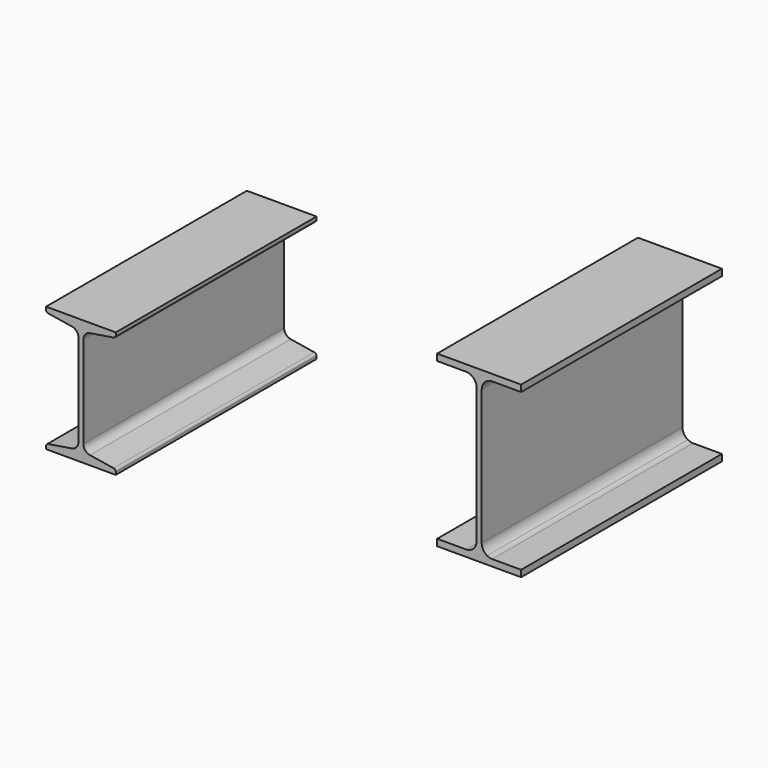
from build123d import *

# Parameters (mm, degrees)
F1_DEPTH = 304.8
F0_W     = 25.4
F0_H     = 4.7064676
F0_H_2   = 4.8951642
F0_H_3   = 5.2649374
F0_H_4   = 6.707251
F0_H_5   = 113.585498
F0_W_2   = 35.433
F0_H_6   = 25.4
F0_H_7   = 5.8125868
F0_H_8   = 115.3748264
F0_H_9   = 6.371082
F0_H_10  = 139.657836
F0_W_3   = 39.37
F4_DEPTH = 304.8
F3_W     = 25.4
F3_H     = 8.7630254
F3_H_2   = 10.9220254
F3_H_3   = 5.461
F3_H_4   = 7.1119746
F3_H_5   = 6.6040508
F3_H_6   = 10.2869492
F3_H_7   = 9.2710254
F3_H_8   = 11.5570508
F3_H_9   = 5.2069492
F3_H_10  = 6.4770254
F3_H_11  = 8.0010508
F3_H_12  = 8.3819492
F3_H_13  = 10.1599238
F3_H_14  = 10.1600508
F3_H_15  = 11.811
F3_H_16  = 11.0490254
F3_H_17  = 12.5730762
F3_H_18  = 181.1020254
F3_H_19  = 12.5729746
F3_H_20  = 14.2240254
F3_H_21  = 14.2239492
F3_H_22  = 17.3990254
F3_H_23  = 181.1020508
F3_H_24  = 17.3989238


# Not quite as in the source:
# - ends of sketch curves that miss each other by under 0.0002 mm in the source are joined


with BuildPart() as f1:
    # F0 (on Front) → F1 (new body)
    with BuildSketch(Plane.XZ):
        with BuildLine():
            Line((-460.2807914, 271.1249848), (-460.2807914, 273.6544184))
            Line((-460.2807914, 273.6544184), (-519.4627914, 273.6544184))
            Line((-519.4627914, 273.6544184), (-519.4627914, 271.1249848))
            ThreePointArc((-519.4627914, 271.1249848), (-518.9356844083, 269.6944587174), (-517.606406124, 268.947956275))
            Line((-517.606406124, 268.947956275), (-496.0408672, 265.4974624))
            ThreePointArc((-496.0408672, 265.4974624), (-493.1694240321, 263.8849236604), (-492.0307914, 260.7947794))
            Line((-492.0307914, 260.7947794), (-492.0307914, 210.3140574))
            ThreePointArc((-492.0307914, 210.3140574), (-493.1694240321, 207.2239131396), (-496.0408665917, 205.611370598))
            Line((-496.0408665917, 205.611370598), (-517.606407, 202.160886))
            ThreePointArc((-517.606407, 202.160886), (-518.9356844083, 201.4143780826), (-519.4627914, 199.983852))
            Line((-519.4627914, 199.983852), (-519.4627914, 197.4544184))
            Line((-519.4627914, 197.4544184), (-489.8717914, 197.4544184))
            Line((-489.8717914, 197.4544184), (-460.2807914, 197.4544184))
            Line((-460.2807914, 197.4544184), (-460.2807914, 199.983852))
            ThreePointArc((-460.2807914, 199.983852), (-460.8078983917, 201.4143780826), (-462.137176676, 202.160880525))
            Line((-462.137176676, 202.160880525), (-483.7027156, 205.6113744))
            ThreePointArc((-483.7027156, 205.6113744), (-486.5741587679, 207.2239131396), (-487.7127914, 210.3140574))
            Line((-487.7127914, 210.3140574), (-487.7127914, 260.7947794))
            ThreePointArc((-487.7127914, 260.7947794), (-486.5741587679, 263.8849236604), (-483.7027162083, 265.497466202))
            Line((-483.7027162083, 265.497466202), (-462.1371758, 268.9479508))
            ThreePointArc((-462.1371758, 268.9479508), (-460.8078983917, 269.6944587174), (-460.2807914, 271.1249848))
        make_face()
    extrude(amount=F1_DEPTH)


with BuildPart() as f1b:
    # F0 (on Front) → F1, piece 2 (new body)
    with BuildSketch(Plane.XZ):
        Polygon((-379.0338114, 197.4544184), (-351.6018114, 197.4544184), (-351.6018114, 222.8544184), (-379.0338114, 222.8544184), (-379.0338114, 199.6134184), align=None)
        Polygon((-381.1928114, 197.4544184), (-379.0338114, 197.4544184), (-379.0338114, 199.6134184), align=None)
        Polygon((-379.0338114, 199.6134184), (-379.0338114, 222.8544184), (-383.3518114, 222.8544184), (-383.3518114, 199.6134184), (-381.1928114, 197.4544184), align=None)
        Polygon((-383.3518114, 197.4544184), (-381.1928114, 197.4544184), (-383.3518114, 199.6134184), align=None)
        Polygon((-383.3518114, 199.6134184), (-383.3518114, 222.8544184), (-410.7838114, 222.8544184), (-410.7838114, 197.4544184), (-383.3518114, 197.4544184), align=None)
    extrude(amount=F1_DEPTH)


with BuildPart() as f1c:
    # F0 (on Front) → F1, piece 3 (new body)
    with BuildSketch(Plane.XZ):
        with Locations((-272.4884314, 271.3011846)):
            Rectangle(F0_W, F0_H)
        Polygon((-259.7884314, 202.160886), (-259.7884314, 268.9479508), (-285.1884314, 268.9479508), (-285.1884314, 202.160886), (-280.4819638, 202.160886), align=None)
        Polygon((-259.7884314, 197.4544184), (-259.7884314, 202.160886), (-280.4819638, 202.160886), (-285.1884314, 197.4544184), align=None)
        Polygon((-285.1884314, 197.4544184), (-280.4819638, 202.160886), (-285.1884314, 202.160886), align=None)
    extrude(amount=F1_DEPTH)


with BuildPart() as f1d:
    # F0 (on Front) → F1, piece 4 (new body)
    with BuildSketch(Plane.XZ):
        with BuildLine():
            Line((-155.3543756, 265.4974624), (-133.7888358, 268.9479508))
            ThreePointArc((-133.7888358, 268.9479508), (-132.4595583917, 269.6944587174), (-131.9324514, 271.1249848))
            Line((-131.9324514, 271.1249848), (-131.9324514, 273.6544184))
            Line((-131.9324514, 273.6544184), (-195.6610514, 273.6544184))
            Line((-195.6610514, 273.6544184), (-195.6610514, 271.1249848))
            ThreePointArc((-195.6610514, 271.1249848), (-195.1339444083, 269.6944587174), (-193.804666124, 268.947956275))
            Line((-193.804666124, 268.947956275), (-172.2391272, 265.4974624))
            ThreePointArc((-172.2391272, 265.4974624), (-169.3676840321, 263.8849236604), (-168.2290514, 260.7947794))
            Line((-168.2290514, 260.7947794), (-168.2290514, 210.3140574))
            ThreePointArc((-168.2290514, 210.3140574), (-169.3676840321, 207.2239131396), (-172.2391265917, 205.611370598))
            Line((-172.2391265917, 205.611370598), (-193.804667, 202.160886))
            ThreePointArc((-193.804667, 202.160886), (-195.1339444083, 201.4143780826), (-195.6610514, 199.983852))
            Line((-195.6610514, 199.983852), (-195.6610514, 197.4544184))
            Line((-195.6610514, 197.4544184), (-163.7967514, 197.4544184))
            Line((-163.7967514, 197.4544184), (-131.9324514, 197.4544184))
            Line((-131.9324514, 197.4544184), (-131.9324514, 199.983852))
            ThreePointArc((-131.9324514, 199.983852), (-132.4595583917, 201.4143780826), (-133.788836676, 202.160880525))
            Line((-133.788836676, 202.160880525), (-155.3543756, 205.6113744))
            ThreePointArc((-155.3543756, 205.6113744), (-158.2258187679, 207.2239131396), (-159.3644514, 210.3140574))
            Line((-159.3644514, 210.3140574), (-159.3644514, 260.7947794))
            ThreePointArc((-159.3644514, 260.7947794), (-158.2258187679, 263.8849236604), (-155.3543756, 265.4974624))
        make_face()
    extrude(amount=F1_DEPTH)


with BuildPart() as f1e:
    # F0 (on Front) → F1, piece 5 (new body)
    with BuildSketch(Plane.XZ):
        Polygon((-50.6727714, 197.4544184), (-23.2407714, 197.4544184), (-23.2407714, 222.8544184), (-50.6727714, 222.8544184), (-50.6727714, 201.8867184), align=None)
        Polygon((-55.1050714, 197.4544184), (-50.6727714, 197.4544184), (-50.6727714, 201.8867184), align=None)
        Polygon((-50.6727714, 201.8867184), (-50.6727714, 222.8544184), (-59.5373714, 222.8544184), (-59.5373714, 201.8867184), (-55.1050714, 197.4544184), align=None)
        Polygon((-59.5373714, 197.4544184), (-55.1050714, 197.4544184), (-59.5373714, 201.8867184), align=None)
        Polygon((-59.5373714, 201.8867184), (-59.5373714, 222.8544184), (-86.9693714, 222.8544184), (-86.9693714, 197.4544184), (-59.5373714, 197.4544184), align=None)
    extrude(amount=F1_DEPTH)


with BuildPart() as f1f:
    # F0 (on Front) → F1, piece 6 (new body)
    with BuildSketch(Plane.XZ):
        with Locations((53.5866086, 271.3011846)):
            Rectangle(F0_W, F0_H)
        Polygon((66.2866086, 202.160886), (66.2866086, 268.9479508), (40.8866086, 268.9479508), (40.8866086, 202.160886), (45.5930762, 202.160886), align=None)
        Polygon((66.2866086, 197.4544184), (66.2866086, 202.160886), (45.5930762, 202.160886), (40.8866086, 197.4544184), align=None)
        Polygon((45.5930762, 202.160886), (40.8866086, 202.160886), (40.8866086, 197.4544184), align=None)
    extrude(amount=F1_DEPTH)


with BuildPart() as f1g:
    # F0 (on Front) → F1, piece 7 (new body)
    with BuildSketch(Plane.XZ):
        with BuildLine():
            Line((200.4290886, 296.4235626), (200.4290886, 299.0544184))
            Line((200.4290886, 299.0544184), (124.1274886, 299.0544184))
            Line((124.1274886, 299.0544184), (124.1274886, 296.4235626))
            ThreePointArc((124.1274886, 296.4235626), (124.6757347672, 294.9356762233), (126.0583196018, 294.1592492112))
            Line((126.0583196018, 294.1592492112), (154.4804378, 289.6117144))
            ThreePointArc((154.4804378, 289.6117144), (158.3090171817, 287.4616563857), (159.8271886, 283.3414704))
            Line((159.8271886, 283.3414704), (159.8271886, 213.1673664))
            ThreePointArc((159.8271886, 213.1673664), (158.3090171817, 209.0471804143), (154.4804381884, 206.8971199724))
            Line((154.4804381884, 206.8971199724), (126.0583204, 202.3495826))
            ThreePointArc((126.0583204, 202.3495826), (124.6757347672, 201.5731605767), (124.1274886, 200.0852742))
            Line((124.1274886, 200.0852742), (124.1274886, 197.4544184))
            Line((124.1274886, 197.4544184), (162.2782886, 197.4544184))
            Line((162.2782886, 197.4544184), (200.4290886, 197.4544184))
            Line((200.4290886, 197.4544184), (200.4290886, 200.0852742))
            ThreePointArc((200.4290886, 200.0852742), (199.8808424328, 201.5731605767), (198.4982575982, 202.3495875888))
            Line((198.4982575982, 202.3495875888), (170.0761394, 206.8971224))
            ThreePointArc((170.0761394, 206.8971224), (166.2475600183, 209.0471804143), (164.7293886, 213.1673664))
            Line((164.7293886, 213.1673664), (164.7293886, 283.3414704))
            ThreePointArc((164.7293886, 283.3414704), (166.2475600183, 287.4616563857), (170.0761390116, 289.6117168276))
            Line((170.0761390116, 289.6117168276), (198.4982568, 294.1592542))
            ThreePointArc((198.4982568, 294.1592542), (199.8808424328, 294.9356762233), (200.4290886, 296.4235626))
        make_face()
    extrude(amount=F1_DEPTH)


with BuildPart() as f1h:
    # F0 (on Front) → F1, piece 8 (new body)
    with BuildSketch(Plane.XZ):
        Polygon((273.4210686, 197.4544184), (309.1207686, 197.4544184), (309.1207686, 222.8544184), (268.5188686, 222.8544184), (268.5188686, 199.9055184), (270.9699686, 197.4544184), (273.4210686, 199.9055184), align=None)
        Polygon((270.9699686, 197.4544184), (273.4210686, 197.4544184), (273.4210686, 199.9055184), align=None)
        Polygon((268.5188686, 199.9055184), (268.5188686, 222.8544184), (232.8191686, 222.8544184), (232.8191686, 197.4544184), (268.5188686, 197.4544184), align=None)
        Polygon((268.5188686, 197.4544184), (270.9699686, 197.4544184), (268.5188686, 199.9055184), align=None)
    extrude(amount=F1_DEPTH)


with BuildPart() as f1i:
    # F0 (on Front) → F1, piece 9 (new body)
    with BuildSketch(Plane.XZ):
        with Locations((379.6616486, 296.6068363)):
            Rectangle(F0_W, F0_H_2)
        Polygon((392.3616486, 202.3495826), (392.3616486, 294.1592542), (366.9616486, 294.1592542), (366.9616486, 202.3495826), (371.8568128, 202.3495826), align=None)
        Polygon((392.3616486, 197.4544184), (392.3616486, 202.3495826), (371.8568128, 202.3495826), (366.9616486, 197.4544184), align=None)
        Polygon((371.8568128, 202.3495826), (366.9616486, 202.3495826), (366.9616486, 197.4544184), align=None)
    extrude(amount=F1_DEPTH)


with BuildPart() as f1j:
    # F0 (on Front) → F1, piece 10 (new body)
    with BuildSketch(Plane.XZ):
        with BuildLine():
            Line((523.8625286, 296.224833), (523.8625286, 299.0544184))
            Line((523.8625286, 299.0544184), (452.8441286, 299.0544184))
            Line((452.8441286, 299.0544184), (452.8441286, 296.224833))
            ThreePointArc((452.8441286, 296.224833), (453.4337860156, 294.6245531891), (454.9208053543, 293.7894694644))
            Line((454.9208053543, 293.7894694644), (478.8663778, 289.9581704))
            ThreePointArc((478.8663778, 289.9581704), (482.6949571817, 287.8081123857), (484.2131286, 283.6879264))
            Line((484.2131286, 283.6879264), (484.2131286, 212.8209104))
            ThreePointArc((484.2131286, 212.8209104), (482.6949571817, 208.7007244143), (478.8663781884, 206.5506639724))
            Line((478.8663781884, 206.5506639724), (454.9208072, 202.7193558))
            ThreePointArc((454.9208072, 202.7193558), (453.4337860156, 201.8842836109), (452.8441286, 200.2840038))
            Line((452.8441286, 200.2840038), (452.8441286, 197.4544184))
            Line((452.8441286, 197.4544184), (488.3533286, 197.4544184))
            Line((488.3533286, 197.4544184), (523.8625286, 197.4544184))
            Line((523.8625286, 197.4544184), (523.8625286, 200.2840038))
            ThreePointArc((523.8625286, 200.2840038), (523.2728711844, 201.8842836109), (521.7858518457, 202.7193673356))
            Line((521.7858518457, 202.7193673356), (497.8402794, 206.5506664))
            ThreePointArc((497.8402794, 206.5506664), (494.0117000183, 208.7007244143), (492.4935286, 212.8209104))
            Line((492.4935286, 212.8209104), (492.4935286, 283.6879264))
            ThreePointArc((492.4935286, 283.6879264), (494.0117000183, 287.8081123857), (497.8402790116, 289.9581728276))
            Line((497.8402790116, 289.9581728276), (521.78585, 293.789481))
            ThreePointArc((521.78585, 293.789481), (523.2728711844, 294.6245531891), (523.8625286, 296.224833))
        make_face()
    extrude(amount=F1_DEPTH)


with BuildPart() as f1k:
    # F0 (on Front) → F1, piece 11 (new body)
    with BuildSketch(Plane.XZ):
        Polygon((-485.7315914, -34.3368376), (-454.3625914, -34.3368376), (-454.3625914, -8.9368376), (-485.7315914, -8.9368376), (-485.7315914, -30.1966376), align=None)
        Polygon((-489.8717914, -34.3368376), (-485.7315914, -34.3368376), (-485.7315914, -30.1966376), align=None)
        Polygon((-485.7315914, -30.1966376), (-485.7315914, -8.9368376), (-494.0119914, -8.9368376), (-494.0119914, -30.1966376), (-489.8717914, -34.3368376), align=None)
        Polygon((-494.0119914, -34.3368376), (-489.8717914, -34.3368376), (-494.0119914, -30.1966376), align=None)
        Polygon((-494.0119914, -30.1966376), (-494.0119914, -8.9368376), (-525.3809914, -8.9368376), (-525.3809914, -34.3368376), (-494.0119914, -34.3368376), align=None)
    extrude(amount=F1_DEPTH)


with BuildPart() as f1l:
    # F0 (on Front) → F1, piece 12 (new body)
    with BuildSketch(Plane.XZ):
        with Locations((-381.1801114, 64.6306937)):
            Rectangle(F0_W, F0_H_3)
        Polygon((-368.4801114, -29.0719002), (-368.4801114, 61.998225), (-393.8801114, 61.998225), (-393.8801114, -29.0719002), (-388.615174, -29.0719002), align=None)
        Polygon((-368.4801114, -34.3368376), (-368.4801114, -29.0719002), (-388.615174, -29.0719002), (-393.8801114, -34.3368376), align=None)
        Polygon((-393.8801114, -34.3368376), (-388.615174, -29.0719002), (-393.8801114, -29.0719002), align=None)
    extrude(amount=F1_DEPTH)


with BuildPart() as f1m:
    # F0 (on Front) → F1, piece 13 (new body)
    with BuildSketch(Plane.XZ):
        with BuildLine():
            Line((-263.0871802, 81.7792624), (-236.9832192, 85.9559114))
            ThreePointArc((-236.9832192, 85.9559114), (-235.0888271575, 87.0197464504), (-234.3376314, 89.0584198))
            Line((-234.3376314, 89.0584198), (-234.3376314, 92.6631624))
            Line((-234.3376314, 92.6631624), (-310.6392314, 92.6631624))
            Line((-310.6392314, 92.6631624), (-310.6392314, 89.0584198))
            ThreePointArc((-310.6392314, 89.0584198), (-309.8880356425, 87.0197464504), (-307.9936454789, 85.9558996568))
            Line((-307.9936454789, 85.9558996568), (-281.8896826, 81.7792624))
            ThreePointArc((-281.8896826, 81.7792624), (-277.1039497413, 79.0916946533), (-275.2062314, 73.9414574))
            Line((-275.2062314, 73.9414574), (-275.2062314, -15.6151326))
            ThreePointArc((-275.2062314, -15.6151326), (-277.1039497413, -20.7653698533), (-281.8896817975, -23.4529426158))
            Line((-281.8896817975, -23.4529426158), (-307.9936436, -27.6295866))
            ThreePointArc((-307.9936436, -27.6295866), (-309.8880356425, -28.6934216504), (-310.6392314, -30.732095))
            Line((-310.6392314, -30.732095), (-310.6392314, -34.3368376))
            Line((-310.6392314, -34.3368376), (-272.4884314, -34.3368376))
            Line((-272.4884314, -34.3368376), (-234.3376314, -34.3368376))
            Line((-234.3376314, -34.3368376), (-234.3376314, -30.732095))
            ThreePointArc((-234.3376314, -30.732095), (-235.0888271575, -28.6934216504), (-236.9832173211, -27.6295748568))
            Line((-236.9832173211, -27.6295748568), (-263.0871802, -23.4529376))
            ThreePointArc((-263.0871802, -23.4529376), (-267.8729130587, -20.7653698533), (-269.7706314, -15.6151326))
            Line((-269.7706314, -15.6151326), (-269.7706314, 73.9414574))
            ThreePointArc((-269.7706314, 73.9414574), (-267.8729130587, 79.0916946533), (-263.0871802, 81.7792624))
        make_face()
    extrude(amount=F1_DEPTH)


with BuildPart() as f1n:
    # F0 (on Front) → F1, piece 14 (new body)
    with BuildSketch(Plane.XZ):
        Polygon((-161.0789514, -34.3368376), (-125.6459514, -34.3368376), (-125.6459514, -8.9368376), (-161.0789514, -8.9368376), (-161.0789514, -31.6190376), align=None)
        Polygon((-163.7967514, -34.3368376), (-161.0789514, -34.3368376), (-161.0789514, -31.6190376), align=None)
        Polygon((-161.0789514, -31.6190376), (-161.0789514, -8.9368376), (-166.5145514, -8.9368376), (-166.5145514, -31.6190376), (-163.7967514, -34.3368376), align=None)
        Polygon((-166.5145514, -34.3368376), (-163.7967514, -34.3368376), (-166.5145514, -31.6190376), align=None)
        Polygon((-166.5145514, -31.6190376), (-166.5145514, -8.9368376), (-201.9475514, -8.9368376), (-201.9475514, -34.3368376), (-166.5145514, -34.3368376), align=None)
    extrude(amount=F1_DEPTH)


with BuildPart() as f1o:
    # F0 (on Front) → F1, piece 15 (new body)
    with BuildSketch(Plane.XZ):
        with Locations((-55.1050714, 89.3095369)):
            Rectangle(F0_W, F0_H_4)
        with Locations((-55.1050714, 29.1631624)):
            Rectangle(F0_W, F0_H_5)
        with Locations((-55.1050714, -30.9832121)):
            Rectangle(F0_W, F0_H_4)
    extrude(amount=F1_DEPTH)


with BuildPart() as f1p:
    # F0 (on Front) → F1, piece 16 (new body)
    with BuildSketch(Plane.XZ):
        with BuildLine():
            Line((95.2934086, 89.5392418), (95.2934086, 92.6631624))
            Line((95.2934086, 92.6631624), (11.8798086, 92.6631624))
            Line((11.8798086, 92.6631624), (11.8798086, 89.5392418))
            ThreePointArc((11.8798086, 89.5392418), (12.5307976686, 87.7725093747), (14.172486546, 86.8505615127))
            Line((14.172486546, 86.8505615127), (40.6293574, 82.6174624))
            ThreePointArc((40.6293574, 82.6174624), (45.4150902587, 79.9298946533), (47.3128086, 74.7796574))
            Line((47.3128086, 74.7796574), (47.3128086, -16.4533326))
            ThreePointArc((47.3128086, -16.4533326), (45.4150902587, -21.6035698533), (40.6293582025, -24.2911426158))
            Line((40.6293582025, -24.2911426158), (14.1724888, -28.5242508))
            ThreePointArc((14.1724888, -28.5242508), (12.5307976686, -29.4461845747), (11.8798086, -31.212917))
            Line((11.8798086, -31.212917), (11.8798086, -34.3368376))
            Line((11.8798086, -34.3368376), (53.5866086, -34.3368376))
            Line((53.5866086, -34.3368376), (95.2934086, -34.3368376))
            Line((95.2934086, -34.3368376), (95.2934086, -31.212917))
            ThreePointArc((95.2934086, -31.212917), (94.6424195314, -29.4461845747), (93.000730654, -28.5242367127))
            Line((93.000730654, -28.5242367127), (66.5438598, -24.2911376))
            ThreePointArc((66.5438598, -24.2911376), (61.7581269413, -21.6035698533), (59.8604086, -16.4533326))
            Line((59.8604086, -16.4533326), (59.8604086, 74.7796574))
            ThreePointArc((59.8604086, 74.7796574), (61.7581269413, 79.9298946533), (66.5438589975, 82.6174674158))
            Line((66.5438589975, 82.6174674158), (93.0007284, 86.8505756))
            ThreePointArc((93.0007284, 86.8505756), (94.6424195314, 87.7725093747), (95.2934086, 89.5392418))
        make_face()
    extrude(amount=F1_DEPTH)


with BuildPart() as f1q:
    # F0 (on Front) → F1, piece 17 (new body)
    with BuildSketch(Plane.XZ):
        with Locations((186.2685886, -21.6368376)):
            Rectangle(F0_W_2, F0_H_6)
        Polygon((162.2782886, -34.3368376), (168.5520886, -34.3368376), (168.5520886, -8.9368376), (156.0044886, -8.9368376), (156.0044886, -34.3368376), align=None)
        with Locations((138.2879886, -21.6368376)):
            Rectangle(F0_W_2, F0_H_6)
    extrude(amount=F1_DEPTH)


with BuildPart() as f1r:
    # F0 (on Front) → F1, piece 18 (new body)
    with BuildSketch(Plane.XZ):
        with Locations((270.9699686, 89.756869)):
            Rectangle(F0_W, F0_H_7)
        with Locations((270.9699686, 29.1631624)):
            Rectangle(F0_W, F0_H_8)
        with Locations((270.9699686, -31.4305442)):
            Rectangle(F0_W, F0_H_7)
    extrude(amount=F1_DEPTH)


with BuildPart() as f1s:
    # F0 (on Front) → F1, piece 19 (new body)
    with BuildSketch(Plane.XZ):
        with BuildLine():
            Line((390.6282002, 107.0781958), (419.4650742, 111.6920804))
            ThreePointArc((419.4650742, 111.6920804), (421.2645078056, 112.7026023195), (421.9780486, 114.63909))
            Line((421.9780486, 114.63909), (421.9780486, 118.0631624))
            Line((421.9780486, 118.0631624), (337.3452486, 118.0631624))
            Line((337.3452486, 118.0631624), (337.3452486, 114.63909))
            ThreePointArc((337.3452486, 114.63909), (338.0587893944, 112.7026023195), (339.8582219869, 111.6920740681))
            Line((339.8582219869, 111.6920740681), (368.695097, 107.0781958))
            ThreePointArc((368.695097, 107.0781958), (374.4379820338, 103.8530944476), (376.7152486, 97.6728044))
            Line((376.7152486, 97.6728044), (376.7152486, -13.9464796))
            ThreePointArc((376.7152486, -13.9464796), (374.4379820338, -20.1267696476), (368.6950942541, -23.351853838))
            Line((368.6950942541, -23.351853838), (339.858223, -27.9657556))
            ThreePointArc((339.858223, -27.9657556), (338.0587893944, -28.9762775195), (337.3452486, -30.9127652))
            Line((337.3452486, -30.9127652), (337.3452486, -34.3368376))
            Line((337.3452486, -34.3368376), (379.6616486, -34.3368376))
            Line((379.6616486, -34.3368376), (421.9780486, -34.3368376))
            Line((421.9780486, -34.3368376), (421.9780486, -30.9127652))
            ThreePointArc((421.9780486, -30.9127652), (421.2645078056, -28.9762775195), (419.4650752131, -27.9657492681))
            Line((419.4650752131, -27.9657492681), (390.6282002, -23.351871))
            ThreePointArc((390.6282002, -23.351871), (384.8853151662, -20.1267696476), (382.6080486, -13.9464796))
            Line((382.6080486, -13.9464796), (382.6080486, 97.6728044))
            ThreePointArc((382.6080486, 97.6728044), (384.8853151662, 103.8530944476), (390.6282002, 107.0781958))
        make_face()
    extrude(amount=F1_DEPTH)


with BuildPart() as f1t:
    # F0 (on Front) → F1, piece 20 (new body)
    with BuildSketch(Plane.XZ):
        Polygon((491.2870286, -34.3368376), (530.6570286, -34.3368376), (530.6570286, -8.9368376), (491.2870286, -8.9368376), (491.2870286, -31.3904376), align=None)
        Polygon((488.3406286, -34.3368376), (491.2870286, -34.3368376), (491.2870286, -31.3904376), align=None)
        Polygon((491.2870286, -31.3904376), (491.2870286, -8.9368376), (485.3942286, -8.9368376), (485.3942286, -31.3904376), (488.3406286, -34.3368376), align=None)
        Polygon((485.3942286, -34.3368376), (488.3406286, -34.3368376), (485.3942286, -31.3904376), align=None)
        Polygon((485.3942286, -31.3904376), (485.3942286, -8.9368376), (446.0242286, -8.9368376), (446.0242286, -34.3368376), (485.3942286, -34.3368376), align=None)
    extrude(amount=F1_DEPTH)


with BuildPart() as f1u:
    # F0 (on Front) → F1, piece 21 (new body)
    with BuildSketch(Plane.XZ):
        with Locations((-489.8717914, -116.9136346)):
            Rectangle(F0_W, F0_H_9)
        with Locations((-489.8717914, -189.9280936)):
            Rectangle(F0_W, F0_H_10)
        with Locations((-489.8717914, -262.9425526)):
            Rectangle(F0_W, F0_H_9)
    extrude(amount=F1_DEPTH)


with BuildPart() as f1v:
    # F0 (on Front) → F1, piece 22 (new body)
    with BuildSketch(Plane.XZ):
        with BuildLine():
            Line((-335.9046114, -117.152166), (-335.9046114, -113.7280936))
            Line((-335.9046114, -113.7280936), (-426.4556114, -113.7280936))
            Line((-426.4556114, -113.7280936), (-426.4556114, -117.152166))
            ThreePointArc((-426.4556114, -117.152166), (-425.7420706056, -119.0886536805), (-423.9426380131, -120.0991819319))
            Line((-423.9426380131, -120.0991819319), (-395.105763, -124.7130602))
            ThreePointArc((-395.105763, -124.7130602), (-389.3628779662, -127.9381615524), (-387.0856114, -134.1184516))
            Line((-387.0856114, -134.1184516), (-387.0856114, -245.7377356))
            ThreePointArc((-387.0856114, -245.7377356), (-389.3628779662, -251.9180256476), (-395.1057657459, -255.143109838))
            Line((-395.1057657459, -255.143109838), (-423.942637, -259.7570116))
            ThreePointArc((-423.942637, -259.7570116), (-425.7420706056, -260.7675335195), (-426.4556114, -262.7040212))
            Line((-426.4556114, -262.7040212), (-426.4556114, -266.1280936))
            Line((-426.4556114, -266.1280936), (-381.1801114, -266.1280936))
            Line((-381.1801114, -266.1280936), (-335.9046114, -266.1280936))
            Line((-335.9046114, -266.1280936), (-335.9046114, -262.7040212))
            ThreePointArc((-335.9046114, -262.7040212), (-336.6181521944, -260.7675335195), (-338.4175847869, -259.7570052681))
            Line((-338.4175847869, -259.7570052681), (-367.2544598, -255.143127))
            ThreePointArc((-367.2544598, -255.143127), (-372.9973448338, -251.9180256476), (-375.2746114, -245.7377356))
            Line((-375.2746114, -245.7377356), (-375.2746114, -134.1184516))
            ThreePointArc((-375.2746114, -134.1184516), (-372.9973448338, -127.9381615524), (-367.2544570541, -124.713077362))
            Line((-367.2544570541, -124.713077362), (-338.4175858, -120.0991756))
            ThreePointArc((-338.4175858, -120.0991756), (-336.6181521944, -119.0886536805), (-335.9046114, -117.152166))
        make_face()
    extrude(amount=F1_DEPTH)


with BuildPart() as f1w:
    # F0 (on Front) → F1, piece 23 (new body)
    with BuildSketch(Plane.XZ):
        with Locations((-246.8979314, -253.4280936)):
            Rectangle(F0_W_3, F0_H_6)
        Polygon((-266.5829314, -266.1280936), (-266.5829314, -240.7280936), (-278.3939314, -240.7280936), (-278.3939314, -266.1280936), (-272.4884314, -266.1280936), align=None)
        with Locations((-298.0789314, -253.4280936)):
            Rectangle(F0_W_3, F0_H_6)
    extrude(amount=F1_DEPTH)


with BuildPart() as f1x:
    # F0 (on Front) → F1, piece 24 (new body)
    with BuildSketch(Plane.XZ):
        with Locations((-163.7967514, -116.9136346)):
            Rectangle(F0_W, F0_H_9)
        with Locations((-163.7967514, -189.9280936)):
            Rectangle(F0_W, F0_H_10)
        with Locations((-163.7967514, -262.9425526)):
            Rectangle(F0_W, F0_H_9)
    extrude(amount=F1_DEPTH)


with BuildPart() as f4:
    # F3 (on Front) → F4 (new body)
    with BuildSketch(Plane.XZ):
        with BuildLine():
            Line((-1413.5770052, 765.8062916), (-1413.5770052, 757.0432916))
            Line((-1413.5770052, 757.0432916), (-1362.0150052, 757.0432916))
            Line((-1362.0150052, 757.0432916), (-1370.9018835071, 765.9301699071))
            ThreePointArc((-1370.9018835071, 765.9301699071), (-1371.5354380261, 765.8373341355), (-1372.1750052, 765.8062916))
            Line((-1372.1750052, 765.8062916), (-1413.5770052, 765.8062916))
        make_face()
        with BuildLine():
            Line((-1353.1281268929, 765.9301699071), (-1362.0150052, 757.0432916))
            Line((-1362.0150052, 757.0432916), (-1310.4530052, 757.0432916))
            Line((-1310.4530052, 757.0432916), (-1310.4530052, 765.8062916))
            Line((-1310.4530052, 765.8062916), (-1351.8550052, 765.8062916))
            ThreePointArc((-1351.8550052, 765.8062916), (-1352.4945723739, 765.8373341355), (-1353.1281268929, 765.9301699071))
        make_face()
        with BuildLine():
            Line((-1370.9018835071, 765.9301699071), (-1362.0150052, 757.0432916))
            Line((-1362.0150052, 757.0432916), (-1353.1281268929, 765.9301699071))
            ThreePointArc((-1353.1281268929, 765.9301699071), (-1356.9550302813, 768.2147510901), (-1358.4590052, 772.4102916))
            Line((-1358.4590052, 772.4102916), (-1358.4590052, 847.3402916))
            ThreePointArc((-1358.4590052, 847.3402916), (-1356.524738383, 852.010024783), (-1351.8550052, 853.9442916))
            Line((-1351.8550052, 853.9442916), (-1310.4530052, 853.9442916))
            Line((-1310.4530052, 853.9442916), (-1310.4530052, 862.7072916))
            Line((-1310.4530052, 862.7072916), (-1413.5770052, 862.7072916))
            Line((-1413.5770052, 862.7072916), (-1413.5770052, 853.9442916))
            Line((-1413.5770052, 853.9442916), (-1372.1750052, 853.9442916))
            ThreePointArc((-1372.1750052, 853.9442916), (-1367.505272017, 852.010024783), (-1365.5710052, 847.3402916))
            Line((-1365.5710052, 847.3402916), (-1365.5710052, 772.4102916))
            ThreePointArc((-1365.5710052, 772.4102916), (-1367.0749801187, 768.2147510901), (-1370.9018835071, 765.9301699071))
        make_face()
    extrude(amount=F4_DEPTH)


with BuildPart() as f4b:
    # F3 (on Front) → F4, piece 2 (new body)
    with BuildSketch(Plane.XZ):
        Polygon((-1111.2179198, 757.0432916), (-1063.2119452, 757.0432916), (-1063.2119452, 782.4432916), (-1111.2179198, 782.4432916), (-1111.2179198, 760.599317), align=None)
        Polygon((-1114.7739452, 757.0432916), (-1111.2179198, 757.0432916), (-1111.2179198, 760.599317), align=None)
        Polygon((-1111.2179198, 760.599317), (-1111.2179198, 782.4432916), (-1118.3299198, 782.4432916), (-1118.3299198, 760.5992662), (-1114.7739452, 757.0432916), align=None)
        Polygon((-1118.3299198, 757.0432916), (-1114.7739452, 757.0432916), (-1118.3299198, 760.5992662), align=None)
        Polygon((-1118.3299198, 760.5992662), (-1118.3299198, 782.4432916), (-1166.3359452, 782.4432916), (-1166.3359452, 757.0432916), (-1118.3299198, 757.0432916), align=None)
    extrude(amount=F4_DEPTH)


with BuildPart() as f4c:
    # F3 (on Front) → F4, piece 3 (new body)
    with BuildSketch(Plane.XZ):
        with Locations((-867.5201852, 858.3511789)):
            Rectangle(F3_W, F3_H)
        Polygon((-854.8201852, 853.9696662), (-880.2201852, 853.9696662), (-880.2201852, 765.8317424), (-871.4571344, 765.8317424), (-854.8201852, 765.8317424), align=None)
        Polygon((-871.4571344, 765.8317424), (-880.2201852, 765.8317424), (-880.2201852, 757.0686916), align=None)
        Polygon((-854.8201852, 757.0686916), (-854.8201852, 765.8317424), (-871.4571344, 765.8317424), (-880.2201852, 757.0686916), align=None)
    extrude(amount=F4_DEPTH)


with BuildPart() as f4d:
    # F3 (on Front) → F4, piece 4 (new body)
    with BuildSketch(Plane.XZ):
        with BuildLine():
            Line((-683.7664252, 766.1872916), (-683.7664252, 757.0432916))
            Line((-683.7664252, 757.0432916), (-620.2664252, 757.0432916))
            Line((-620.2664252, 757.0432916), (-629.58951382, 766.36638022))
            ThreePointArc((-629.58951382, 766.36638022), (-630.4238929321, 766.232190488), (-631.2678002, 766.1872916))
            Line((-631.2678002, 766.1872916), (-683.7664252, 766.1872916))
        make_face()
        with BuildLine():
            Line((-610.94333658, 766.36638022), (-620.2664252, 757.0432916))
            Line((-620.2664252, 757.0432916), (-556.7664252, 757.0432916))
            Line((-556.7664252, 757.0432916), (-556.7664252, 766.1872916))
            Line((-556.7664252, 766.1872916), (-609.2650502, 766.1872916))
            ThreePointArc((-609.2650502, 766.1872916), (-610.1089574679, 766.232190488), (-610.94333658, 766.36638022))
        make_face()
        with BuildLine():
            Line((-629.58951382, 766.36638022), (-620.2664252, 757.0432916))
            Line((-620.2664252, 757.0432916), (-610.94333658, 766.36638022))
            ThreePointArc((-610.94333658, 766.36638022), (-615.4539198394, 769.1452620642), (-617.2184252, 774.1406666))
            Line((-617.2184252, 774.1406666), (-617.2184252, 867.1999166))
            ThreePointArc((-617.2184252, 867.1999166), (-614.8889355958, 872.8238019958), (-609.2650502, 875.1532916))
            Line((-609.2650502, 875.1532916), (-556.7664252, 875.1532916))
            Line((-556.7664252, 875.1532916), (-556.7664252, 884.2972916))
            Line((-556.7664252, 884.2972916), (-683.7664252, 884.2972916))
            Line((-683.7664252, 884.2972916), (-683.7664252, 875.1532916))
            Line((-683.7664252, 875.1532916), (-631.2678002, 875.1532916))
            ThreePointArc((-631.2678002, 875.1532916), (-625.6439148042, 872.8238019958), (-623.3144252, 867.1999166))
            Line((-623.3144252, 867.1999166), (-623.3144252, 774.1406666))
            ThreePointArc((-623.3144252, 774.1406666), (-625.0789305606, 769.1452620642), (-629.58951382, 766.36638022))
        make_face()
    extrude(amount=F4_DEPTH)


with BuildPart() as f4e:
    # F3 (on Front) → F4, piece 5 (new body)
    with BuildSketch(Plane.XZ):
        Polygon((-369.9646652, 757.0432916), (-309.5126652, 757.0432916), (-309.5126652, 782.4432916), (-369.9646652, 782.4432916), (-369.9646652, 760.0912916), align=None)
        Polygon((-373.0126652, 757.0432916), (-369.9646652, 757.0432916), (-369.9646652, 760.0912916), align=None)
        Polygon((-369.9646652, 760.0912916), (-369.9646652, 782.4432916), (-376.0606652, 782.4432916), (-376.0606652, 760.0912916), (-373.0126652, 757.0432916), align=None)
        Polygon((-376.0606652, 757.0432916), (-373.0126652, 757.0432916), (-376.0606652, 760.0912916), align=None)
        Polygon((-376.0606652, 760.0912916), (-376.0606652, 782.4432916), (-436.5126652, 782.4432916), (-436.5126652, 757.0432916), (-376.0606652, 757.0432916), align=None)
    extrude(amount=F4_DEPTH)


with BuildPart() as f4f:
    # F3 (on Front) → F4, piece 6 (new body)
    with BuildSketch(Plane.XZ):
        Polygon((-113.0462052, 875.178717), (-138.4462052, 875.178717), (-138.4462052, 766.2126916), (-129.3022052, 766.2126916), (-113.0462052, 766.2126916), align=None)
        Polygon((-129.3022052, 766.2126916), (-138.4462052, 766.2126916), (-138.4462052, 757.0686916), align=None)
        Polygon((-113.0462052, 757.0686916), (-113.0462052, 766.2126916), (-129.3022052, 766.2126916), (-138.4462052, 757.0686916), align=None)
    extrude(amount=F4_DEPTH)


with BuildPart() as f4g:
    # F3 (on Front) → F4, piece 7 (new body)
    with BuildSketch(Plane.XZ):
        with BuildLine():
            Line((57.6138548, 767.9652916), (57.6138548, 757.0432916))
            Line((57.6138548, 757.0432916), (121.4948548, 757.0432916))
            Line((121.4948548, 757.0432916), (110.5464743781, 767.9916720219))
            ThreePointArc((110.5464743781, 767.9916720219), (110.2186170992, 767.9718893677), (109.8902298, 767.9652916))
            Line((109.8902298, 767.9652916), (57.6138548, 767.9652916))
        make_face()
        with BuildLine():
            Line((132.4432352219, 767.9916720219), (121.4948548, 757.0432916))
            Line((121.4948548, 757.0432916), (185.3758548, 757.0432916))
            Line((185.3758548, 757.0432916), (185.3758548, 767.9652916))
            Line((185.3758548, 767.9652916), (133.0994798, 767.9652916))
            ThreePointArc((133.0994798, 767.9652916), (132.7710925008, 767.9718893677), (132.4432352219, 767.9916720219))
        make_face()
        with BuildLine():
            Line((110.5464743781, 767.9916720219), (121.4948548, 757.0432916))
            Line((121.4948548, 757.0432916), (132.4432352219, 767.9916720219))
            ThreePointArc((132.4432352219, 767.9916720219), (127.0909003622, 770.5967469344), (124.9238548, 776.1409166))
            Line((124.9238548, 776.1409166), (124.9238548, 868.7556666))
            ThreePointArc((124.9238548, 868.7556666), (127.3184399221, 874.5367064779), (133.0994798, 876.9312916))
            Line((133.0994798, 876.9312916), (185.3758548, 876.9312916))
            Line((185.3758548, 876.9312916), (185.3758548, 887.8532916))
            Line((185.3758548, 887.8532916), (57.6138548, 887.8532916))
            Line((57.6138548, 887.8532916), (57.6138548, 876.9312916))
            Line((57.6138548, 876.9312916), (109.8902298, 876.9312916))
            ThreePointArc((109.8902298, 876.9312916), (115.6712696779, 874.5367064779), (118.0658548, 868.7556666))
            Line((118.0658548, 868.7556666), (118.0658548, 776.1409166))
            ThreePointArc((118.0658548, 776.1409166), (115.8988092378, 770.5967469344), (110.5464743781, 767.9916720219))
        make_face()
    extrude(amount=F4_DEPTH)


with BuildPart() as f4h:
    # F3 (on Front) → F4, piece 8 (new body)
    with BuildSketch(Plane.XZ):
        Polygon((372.2030148, 757.0686916), (432.6550148, 757.0686916), (432.6550148, 782.4686916), (372.2030148, 782.4686916), (372.2030148, 760.4976916), align=None)
        Polygon((368.7740148, 757.0686916), (372.2030148, 757.0686916), (372.2030148, 760.4976916), align=None)
        Polygon((372.2030148, 760.4976916), (372.2030148, 782.4686916), (365.3450148, 782.4686916), (365.3450148, 760.4976916), (368.7740148, 757.0686916), align=None)
        Polygon((365.3450148, 757.0686916), (368.7740148, 757.0686916), (365.3450148, 760.4976916), align=None)
        Polygon((365.3450148, 760.4976916), (365.3450148, 782.4686916), (304.8930148, 782.4686916), (304.8930148, 757.0686916), (365.3450148, 757.0686916), align=None)
    extrude(amount=F4_DEPTH)


with BuildPart() as f4i:
    # F3 (on Front) → F4, piece 9 (new body)
    with BuildSketch(Plane.XZ):
        Polygon((603.3277748, 876.931317), (603.3277748, 767.965317), (614.2498002, 767.965317), (628.7277748, 767.965317), (628.7277748, 876.931317), align=None)
        Polygon((614.2498002, 767.965317), (603.3277748, 767.965317), (603.3277748, 757.0432916), align=None)
        Polygon((628.7277748, 767.965317), (614.2498002, 767.965317), (603.3277748, 757.0432916), (628.7277748, 757.0432916), align=None)
        with Locations((616.0277748, 882.3923297)):
            Rectangle(F3_W, F3_H_2)
    extrude(amount=F4_DEPTH)


with BuildPart() as f4j:
    # F3 (on Front) → F4, piece 10 (new body)
    with BuildSketch(Plane.XZ):
        with BuildLine():
            Line((813.2181348, 762.5042916), (813.2181348, 757.0432916))
            Line((813.2181348, 757.0432916), (863.2561348, 757.0432916))
            Line((863.2561348, 757.0432916), (856.4937384412, 763.8056879588))
            ThreePointArc((856.4937384412, 763.8056879588), (854.1996095361, 762.8354966505), (851.7308848, 762.5042916))
            Line((851.7308848, 762.5042916), (813.2181348, 762.5042916))
        make_face()
        with BuildLine():
            Line((870.0185311588, 763.8056879588), (863.2561348, 757.0432916))
            Line((863.2561348, 757.0432916), (913.2941348, 757.0432916))
            Line((913.2941348, 757.0432916), (913.2941348, 762.5042916))
            Line((913.2941348, 762.5042916), (874.7813848, 762.5042916))
            ThreePointArc((874.7813848, 762.5042916), (872.3126600639, 762.8354966505), (870.0185311588, 763.8056879588))
        make_face()
        with BuildLine():
            Line((856.4937384412, 763.8056879588), (863.2561348, 757.0432916))
            Line((863.2561348, 757.0432916), (870.0185311588, 763.8056879588))
            ThreePointArc((870.0185311588, 763.8056879588), (866.6469912461, 767.2274520496), (865.4151348, 771.8705416))
            Line((865.4151348, 771.8705416), (865.4151348, 892.0760416))
            ThreePointArc((865.4151348, 892.0760416), (868.1584459107, 898.6989804893), (874.7813848, 901.4422916))
            Line((874.7813848, 901.4422916), (913.2941348, 901.4422916))
            Line((913.2941348, 901.4422916), (913.2941348, 906.9032916))
            Line((913.2941348, 906.9032916), (813.2181348, 906.9032916))
            Line((813.2181348, 906.9032916), (813.2181348, 901.4422916))
            Line((813.2181348, 901.4422916), (851.7308848, 901.4422916))
            ThreePointArc((851.7308848, 901.4422916), (858.3538236893, 898.6989804893), (861.0971348, 892.0760416))
            Line((861.0971348, 892.0760416), (861.0971348, 771.8705416))
            ThreePointArc((861.0971348, 771.8705416), (859.8652783539, 767.2274520496), (856.4937384412, 763.8056879588))
        make_face()
    extrude(amount=F4_DEPTH)


with BuildPart() as f4k:
    # F3 (on Front) → F4, piece 11 (new body)
    with BuildSketch(Plane.XZ):
        Polygon((1112.6688694, 757.0686916), (1160.5478948, 757.0686916), (1160.5478948, 782.4686916), (1112.6688694, 782.4686916), (1112.6688694, 759.2276662), align=None)
        Polygon((1110.5098948, 757.0686916), (1112.6688694, 757.0686916), (1112.6688694, 759.2276662), align=None)
        Polygon((1112.6688694, 759.2276662), (1112.6688694, 782.4686916), (1108.3508694, 782.4686916), (1108.3508694, 759.227717), (1110.5098948, 757.0686916), align=None)
        Polygon((1108.3508694, 757.0686916), (1110.5098948, 757.0686916), (1108.3508694, 759.227717), align=None)
        Polygon((1108.3508694, 759.227717), (1108.3508694, 782.4686916), (1060.4718694, 782.4686916), (1060.4718694, 757.0686916), (1108.3508694, 757.0686916), align=None)
    extrude(amount=F4_DEPTH)


with BuildPart() as f4l:
    # F3 (on Front) → F4, piece 12 (new body)
    with BuildSketch(Plane.XZ):
        with Locations((1357.7763548, 904.1728424)):
            Rectangle(F3_W, F3_H_3)
        Polygon((1370.4763548, 901.4423424), (1345.0763548, 901.4423424), (1345.0763548, 762.5042916), (1350.5373548, 762.5042916), (1370.4763548, 762.5042916), align=None)
        Polygon((1350.5373548, 762.5042916), (1345.0763548, 762.5042916), (1345.0763548, 757.0432916), align=None)
        Polygon((1370.4763548, 757.0432916), (1370.4763548, 762.5042916), (1350.5373548, 762.5042916), (1345.0763548, 757.0432916), align=None)
    extrude(amount=F4_DEPTH)


with BuildPart() as f4m:
    # F3 (on Front) → F4, piece 13 (new body)
    with BuildSketch(Plane.XZ):
        with BuildLine():
            Line((-1364.9233052, 523.1764746), (-1364.9233052, 403.3837246))
            ThreePointArc((-1364.9233052, 403.3837246), (-1366.3354041937, 398.3796298076), (-1370.15509161, 394.85188601))
            Line((-1370.15509161, 394.85188601), (-1362.0023052, 386.6990996))
            Line((-1362.0023052, 386.6990996), (-1353.84951879, 394.85188601))
            ThreePointArc((-1353.84951879, 394.85188601), (-1357.6692062063, 398.3796298076), (-1359.0813052, 403.3837246))
            Line((-1359.0813052, 403.3837246), (-1359.0813052, 523.1764746))
            ThreePointArc((-1359.0813052, 523.1764746), (-1356.2775482513, 529.9453426513), (-1349.5086802, 532.7490996))
            Line((-1349.5086802, 532.7490996), (-1311.2023052, 532.7490996))
            Line((-1311.2023052, 532.7490996), (-1311.2023052, 539.8610996))
            Line((-1311.2023052, 539.8610996), (-1412.8023052, 539.8610996))
            Line((-1412.8023052, 539.8610996), (-1412.8023052, 532.7490996))
            Line((-1412.8023052, 532.7490996), (-1374.4959302, 532.7490996))
            ThreePointArc((-1374.4959302, 532.7490996), (-1367.7270621487, 529.9453426513), (-1364.9233052, 523.1764746))
        make_face()
        with BuildLine():
            Line((-1362.0023052, 386.6990996), (-1370.15509161, 394.85188601))
            ThreePointArc((-1370.15509161, 394.85188601), (-1372.2639962843, 394.0749319615), (-1374.4959302, 393.8110996))
            Line((-1374.4959302, 393.8110996), (-1412.8023052, 393.8110996))
            Line((-1412.8023052, 393.8110996), (-1412.8023052, 386.6990996))
            Line((-1412.8023052, 386.6990996), (-1362.0023052, 386.6990996))
        make_face()
        with BuildLine():
            Line((-1353.84951879, 394.85188601), (-1362.0023052, 386.6990996))
            Line((-1362.0023052, 386.6990996), (-1311.2023052, 386.6990996))
            Line((-1311.2023052, 386.6990996), (-1311.2023052, 393.8110996))
            Line((-1311.2023052, 393.8110996), (-1349.5086802, 393.8110996))
            ThreePointArc((-1349.5086802, 393.8110996), (-1351.7406141157, 394.0749319615), (-1353.84951879, 394.85188601))
        make_face()
    extrude(amount=F4_DEPTH)


with BuildPart() as f4n:
    # F3 (on Front) → F4, piece 14 (new body)
    with BuildSketch(Plane.XZ):
        Polygon((-1111.8402198, 386.7244996), (-1064.7232452, 386.7244996), (-1064.7232452, 412.1244996), (-1111.8402198, 412.1244996), (-1111.8402198, 389.645525), align=None)
        Polygon((-1114.7612452, 386.7244996), (-1111.8402198, 386.7244996), (-1111.8402198, 389.645525), align=None)
        Polygon((-1111.8402198, 389.645525), (-1111.8402198, 412.1244996), (-1117.6822706, 412.1244996), (-1117.6822706, 389.645525), (-1114.7612452, 386.7244996), align=None)
        Polygon((-1117.6822706, 386.7244996), (-1114.7612452, 386.7244996), (-1117.6822706, 389.645525), align=None)
        Polygon((-1117.6822706, 389.645525), (-1117.6822706, 412.1244996), (-1164.7992452, 412.1244996), (-1164.7992452, 386.7244996), (-1117.6822706, 386.7244996), align=None)
    extrude(amount=F4_DEPTH)


with BuildPart() as f4o:
    # F3 (on Front) → F4, piece 15 (new body)
    with BuildSketch(Plane.XZ):
        with Locations((-867.5074852, 543.1630869)):
            Rectangle(F3_W, F3_H_4)
        Polygon((-854.8074852, 539.6070996), (-880.2074852, 539.6070996), (-880.2074852, 393.8110742), (-873.0955106, 393.8110742), (-854.8074852, 393.8110742), align=None)
        Polygon((-873.0955106, 393.8110742), (-880.2074852, 393.8110742), (-880.2074852, 386.6990996), align=None)
        Polygon((-854.8074852, 386.6990996), (-854.8074852, 393.8110742), (-873.0955106, 393.8110742), (-880.2074852, 386.6990996), align=None)
    extrude(amount=F4_DEPTH)


with BuildPart() as f4p:
    # F3 (on Front) → F4, piece 16 (new body)
    with BuildSketch(Plane.XZ):
        with BuildLine():
            Line((-696.3267252, 393.3030996), (-696.3267252, 386.6990996))
            Line((-696.3267252, 386.6990996), (-620.2537252, 386.6990996))
            Line((-620.2537252, 386.6990996), (-628.0584647918, 394.5038391918))
            ThreePointArc((-628.0584647918, 394.5038391918), (-630.2945006158, 393.6081783794), (-632.6838502, 393.3030996))
            Line((-632.6838502, 393.3030996), (-696.3267252, 393.3030996))
        make_face()
        with BuildLine():
            Line((-612.4489856082, 394.5038391918), (-620.2537252, 386.6990996))
            Line((-620.2537252, 386.6990996), (-544.1807252, 386.6990996))
            Line((-544.1807252, 386.6990996), (-544.1807252, 393.3030996))
            Line((-544.1807252, 393.3030996), (-607.8236002, 393.3030996))
            ThreePointArc((-607.8236002, 393.3030996), (-610.2129497842, 393.6081783794), (-612.4489856082, 394.5038391918))
        make_face()
        with BuildLine():
            Line((-628.0584647918, 394.5038391918), (-620.2537252, 386.6990996))
            Line((-620.2537252, 386.6990996), (-612.4489856082, 394.5038391918))
            ThreePointArc((-612.4489856082, 394.5038391918), (-616.0213689905, 397.9935063967), (-617.3327252, 402.8122246))
            Line((-617.3327252, 402.8122246), (-617.3327252, 522.7319746))
            ThreePointArc((-617.3327252, 522.7319746), (-614.5475669707, 529.4559413707), (-607.8236002, 532.2410996))
            Line((-607.8236002, 532.2410996), (-544.1807252, 532.2410996))
            Line((-544.1807252, 532.2410996), (-544.1807252, 538.8450996))
            Line((-544.1807252, 538.8450996), (-696.3267252, 538.8450996))
            Line((-696.3267252, 538.8450996), (-696.3267252, 532.2410996))
            Line((-696.3267252, 532.2410996), (-632.6838502, 532.2410996))
            ThreePointArc((-632.6838502, 532.2410996), (-625.9598834293, 529.4559413707), (-623.1747252, 522.7319746))
            Line((-623.1747252, 522.7319746), (-623.1747252, 402.8122246))
            ThreePointArc((-623.1747252, 402.8122246), (-624.4860814095, 397.9935063967), (-628.0584647918, 394.5038391918))
        make_face()
    extrude(amount=F4_DEPTH)


with BuildPart() as f4q:
    # F3 (on Front) → F4, piece 17 (new body)
    with BuildSketch(Plane.XZ):
        Polygon((-370.0789652, 386.7244996), (-296.9269652, 386.7244996), (-296.9269652, 412.1244996), (-370.0789652, 412.1244996), (-370.0789652, 389.6454996), align=None)
        Polygon((-372.9999652, 386.7244996), (-370.0789652, 386.7244996), (-370.0789652, 389.6454996), align=None)
        Polygon((-370.0789652, 389.6454996), (-370.0789652, 412.1244996), (-375.9209906, 412.1244996), (-375.9209906, 389.645525), (-372.9999652, 386.7244996), align=None)
        Polygon((-375.9209906, 386.7244996), (-372.9999652, 386.7244996), (-375.9209906, 389.645525), align=None)
        Polygon((-375.9209906, 389.645525), (-375.9209906, 412.1244996), (-449.0729652, 412.1244996), (-449.0729652, 386.7244996), (-375.9209906, 386.7244996), align=None)
    extrude(amount=F4_DEPTH)


with BuildPart() as f4r:
    # F3 (on Front) → F4, piece 18 (new body)
    with BuildSketch(Plane.XZ):
        with Locations((-125.7335052, 535.5430996)):
            Rectangle(F3_W, F3_H_5)
        Polygon((-113.0335052, 393.3030488), (-113.0335052, 532.2410742), (-138.4335052, 532.2410742), (-138.4335052, 393.3030488), (-131.829556, 393.3030488), align=None)
        Polygon((-113.0335052, 386.6990996), (-113.0335052, 393.3030488), (-131.829556, 393.3030488), (-138.4335052, 386.6990996), align=None)
        Polygon((-131.829556, 393.3030488), (-138.4335052, 393.3030488), (-138.4335052, 386.6990996), align=None)
    extrude(amount=F4_DEPTH)


with BuildPart() as f4s:
    # F3 (on Front) → F4, piece 19 (new body)
    with BuildSketch(Plane.XZ):
        with BuildLine():
            Line((70.3138548, 396.9860996), (70.3138548, 386.6990996))
            Line((70.3138548, 386.6990996), (121.4948548, 386.6990996))
            Line((121.4948548, 386.6990996), (110.8544084149, 397.3395459851))
            ThreePointArc((110.8544084149, 397.3395459851), (109.5506987147, 397.0748562888), (108.2233548, 396.9860996))
            Line((108.2233548, 396.9860996), (70.3138548, 396.9860996))
        make_face()
        with BuildLine():
            Line((132.1353011851, 397.3395459851), (121.4948548, 386.6990996))
            Line((121.4948548, 386.6990996), (172.6758548, 386.6990996))
            Line((172.6758548, 386.6990996), (172.6758548, 396.9860996))
            Line((172.6758548, 396.9860996), (134.7663548, 396.9860996))
            ThreePointArc((134.7663548, 396.9860996), (133.4390108853, 397.0748562888), (132.1353011851, 397.3395459851))
        make_face()
        with BuildLine():
            Line((110.8544084149, 397.3395459851), (121.4948548, 386.6990996))
            Line((121.4948548, 386.6990996), (132.1353011851, 397.3395459851))
            ThreePointArc((132.1353011851, 397.3395459851), (126.8410403184, 400.9074328845), (124.7968548, 406.9555996))
            Line((124.7968548, 406.9555996), (124.7968548, 525.9545996))
            ThreePointArc((124.7968548, 525.9545996), (127.716853745, 533.004100655), (134.7663548, 535.9240996))
            Line((134.7663548, 535.9240996), (172.6758548, 535.9240996))
            Line((172.6758548, 535.9240996), (172.6758548, 546.2110996))
            Line((172.6758548, 546.2110996), (70.3138548, 546.2110996))
            Line((70.3138548, 546.2110996), (70.3138548, 535.9240996))
            Line((70.3138548, 535.9240996), (108.2233548, 535.9240996))
            ThreePointArc((108.2233548, 535.9240996), (115.272855855, 533.004100655), (118.1928548, 525.9545996))
            Line((118.1928548, 525.9545996), (118.1928548, 406.9555996))
            ThreePointArc((118.1928548, 406.9555996), (116.1486692816, 400.9074328845), (110.8544084149, 397.3395459851))
        make_face()
    extrude(amount=F4_DEPTH)


with BuildPart() as f4t:
    # F3 (on Front) → F4, piece 20 (new body)
    with BuildSketch(Plane.XZ):
        Polygon((372.0760402, 386.7244996), (419.9549894, 386.7244996), (419.9549894, 412.1244996), (372.0760402, 412.1244996), (372.0760402, 390.026525), align=None)
        Polygon((368.7740148, 386.7244996), (372.0760402, 386.7244996), (372.0760402, 390.026525), align=None)
        Polygon((372.0760402, 390.026525), (372.0760402, 412.1244996), (365.471964, 412.1244996), (365.471964, 390.0265504), (368.7740148, 386.7244996), align=None)
        Polygon((365.471964, 386.7244996), (368.7740148, 386.7244996), (365.471964, 390.0265504), align=None)
        Polygon((365.471964, 390.0265504), (365.471964, 412.1244996), (317.5930148, 412.1244996), (317.5930148, 386.7244996), (365.471964, 386.7244996), align=None)
    extrude(amount=F4_DEPTH)


with BuildPart() as f4u:
    # F3 (on Front) → F4, piece 21 (new body)
    with BuildSketch(Plane.XZ):
        with Locations((616.0150748, 541.0675742)):
            Rectangle(F3_W, F3_H_6)
        Polygon((628.7150748, 396.9860488), (628.7150748, 535.9240996), (603.3150748, 535.9240996), (603.3150748, 396.9860488), (613.602024, 396.9860488), align=None)
        Polygon((628.7150748, 386.6990996), (628.7150748, 396.9860488), (613.602024, 396.9860488), (603.3150748, 386.6990996), align=None)
        Polygon((613.602024, 396.9860488), (603.3150748, 396.9860488), (603.3150748, 386.6990996), align=None)
    extrude(amount=F4_DEPTH)


with BuildPart() as f4v:
    # F3 (on Front) → F4, piece 22 (new body)
    with BuildSketch(Plane.XZ):
        with BuildLine():
            Line((786.8148348, 395.9700996), (786.8148348, 386.6990996))
            Line((786.8148348, 386.6990996), (863.2688348, 386.6990996))
            Line((863.2688348, 386.6990996), (853.4271365166, 396.5407978834))
            ThreePointArc((853.4271365166, 396.5407978834), (851.8002073869, 396.1138235266), (850.1243348, 395.9700996))
            Line((850.1243348, 395.9700996), (786.8148348, 395.9700996))
        make_face()
        with BuildLine():
            Line((873.1105330834, 396.5407978834), (863.2688348, 386.6990996))
            Line((863.2688348, 386.6990996), (939.7228348, 386.6990996))
            Line((939.7228348, 386.6990996), (939.7228348, 395.9700996))
            Line((939.7228348, 395.9700996), (876.4133348, 395.9700996))
            ThreePointArc((876.4133348, 395.9700996), (874.7374622131, 396.1138235266), (873.1105330834, 396.5407978834))
        make_face()
        with BuildLine():
            Line((853.4271365166, 396.5407978834), (863.2688348, 386.6990996))
            Line((863.2688348, 386.6990996), (873.1105330834, 396.5407978834))
            ThreePointArc((873.1105330834, 396.5407978834), (868.3702435987, 400.1395501398), (866.5708348, 405.8125996))
            Line((866.5708348, 405.8125996), (866.5708348, 525.0655996))
            ThreePointArc((866.5708348, 525.0655996), (869.4536363062, 532.0252980938), (876.4133348, 534.9080996))
            Line((876.4133348, 534.9080996), (939.7228348, 534.9080996))
            Line((939.7228348, 534.9080996), (939.7228348, 544.1790996))
            Line((939.7228348, 544.1790996), (786.8148348, 544.1790996))
            Line((786.8148348, 544.1790996), (786.8148348, 534.9080996))
            Line((786.8148348, 534.9080996), (850.1243348, 534.9080996))
            ThreePointArc((850.1243348, 534.9080996), (857.0840332938, 532.0252980938), (859.9668348, 525.0655996))
            Line((859.9668348, 525.0655996), (859.9668348, 405.8125996))
            ThreePointArc((859.9668348, 405.8125996), (858.1674260013, 400.1395501398), (853.4271365166, 396.5407978834))
        make_face()
    extrude(amount=F4_DEPTH)


with BuildPart() as f4w:
    # F3 (on Front) → F4, piece 23 (new body)
    with BuildSketch(Plane.XZ):
        Polygon((1186.5829202, 386.7244996), (1186.5829202, 412.1244996), (1113.8118694, 412.1244996), (1113.8118694, 390.0264742), (1113.8118694, 386.7244996), align=None)
        Polygon((1113.8118694, 390.0264742), (1113.8118694, 412.1244996), (1107.2079202, 412.1244996), (1107.2079202, 390.0264742), (1110.5098948, 386.7244996), align=None)
        Polygon((1107.2079202, 390.0264742), (1107.2079202, 412.1244996), (1034.4368694, 412.1244996), (1034.4368694, 386.7244996), (1107.2079202, 386.7244996), align=None)
        Polygon((1113.8118694, 386.7244996), (1113.8118694, 390.0264742), (1110.5098948, 386.7244996), align=None)
        Polygon((1110.5098948, 386.7244996), (1107.2079202, 390.0264742), (1107.2079202, 386.7244996), align=None)
    extrude(amount=F4_DEPTH)


with BuildPart() as f4x:
    # F3 (on Front) → F4, piece 24 (new body)
    with BuildSketch(Plane.XZ):
        Polygon((1345.0636548, 386.6990996), (1370.4636548, 386.6990996), (1370.4636548, 395.970125), (1354.3346802, 395.970125), align=None)
        Polygon((1354.3346802, 395.970125), (1370.4636548, 395.970125), (1370.4636548, 534.9080742), (1345.0636548, 534.9080742), (1345.0636548, 395.970125), align=None)
        Polygon((1345.0636548, 395.970125), (1345.0636548, 386.6990996), (1354.3346802, 395.970125), align=None)
        with Locations((1357.7636548, 539.5435869)):
            Rectangle(F3_W, F3_H_7)
    extrude(amount=F4_DEPTH)


with BuildPart() as f4y:
    # F3 (on Front) → F4, piece 25 (new body)
    with BuildSketch(Plane.XZ):
        with BuildLine():
            Line((-1439.2437052, 27.9119076), (-1439.2437052, 16.3549076))
            Line((-1439.2437052, 16.3549076), (-1362.0277052, 16.3549076))
            Line((-1362.0277052, 16.3549076), (-1373.8628118797, 28.1900142797))
            ThreePointArc((-1373.8628118797, 28.1900142797), (-1375.033208812, 27.9816745596), (-1376.2199552, 27.9119076))
            Line((-1376.2199552, 27.9119076), (-1439.2437052, 27.9119076))
        make_face()
        with BuildLine():
            Line((-1350.1925985203, 28.1900142797), (-1362.0277052, 16.3549076))
            Line((-1362.0277052, 16.3549076), (-1284.8117052, 16.3549076))
            Line((-1284.8117052, 16.3549076), (-1284.8117052, 27.9119076))
            Line((-1284.8117052, 27.9119076), (-1347.8354552, 27.9119076))
            ThreePointArc((-1347.8354552, 27.9119076), (-1349.022201588, 27.9816745596), (-1350.1925985203, 28.1900142797))
        make_face()
        with BuildLine():
            Line((-1373.8628118797, 28.1900142797), (-1362.0277052, 16.3549076))
            Line((-1362.0277052, 16.3549076), (-1350.1925985203, 28.1900142797))
            ThreePointArc((-1350.1925985203, 28.1900142797), (-1355.7870331848, 31.7668924522), (-1357.9637052, 38.0401576))
            Line((-1357.9637052, 38.0401576), (-1357.9637052, 156.7216576))
            ThreePointArc((-1357.9637052, 156.7216576), (-1354.9972094566, 163.8834118566), (-1347.8354552, 166.8499076))
            Line((-1347.8354552, 166.8499076), (-1284.8117052, 166.8499076))
            Line((-1284.8117052, 166.8499076), (-1284.8117052, 178.4069076))
            Line((-1284.8117052, 178.4069076), (-1439.2437052, 178.4069076))
            Line((-1439.2437052, 178.4069076), (-1439.2437052, 166.8499076))
            Line((-1439.2437052, 166.8499076), (-1376.2199552, 166.8499076))
            ThreePointArc((-1376.2199552, 166.8499076), (-1369.0582009434, 163.8834118566), (-1366.0917052, 156.7216576))
            Line((-1366.0917052, 156.7216576), (-1366.0917052, 38.0401576))
            ThreePointArc((-1366.0917052, 38.0401576), (-1368.2683772152, 31.7668924522), (-1373.8628118797, 28.1900142797))
        make_face()
    extrude(amount=F4_DEPTH)


with BuildPart() as f4z:
    # F3 (on Front) → F4, piece 26 (new body)
    with BuildSketch(Plane.XZ):
        Polygon((-1037.5452706, 16.3803076), (-1037.5452706, 41.7803076), (-1110.6971944, 41.7803076), (-1110.6971944, 20.4443584), (-1110.6971944, 16.3803076), align=None)
        Polygon((-1110.6971944, 20.4443584), (-1110.6971944, 41.7803076), (-1118.8251944, 41.7803076), (-1118.8251944, 20.4442568), (-1114.7612452, 16.3803076), align=None)
        Polygon((-1118.8251944, 20.4442568), (-1118.8251944, 41.7803076), (-1191.9772198, 41.7803076), (-1191.9772198, 16.3803076), (-1118.8251944, 16.3803076), align=None)
        Polygon((-1110.6971944, 16.3803076), (-1110.6971944, 20.4443584), (-1114.7612452, 16.3803076), align=None)
        Polygon((-1114.7612452, 16.3803076), (-1118.8251944, 20.4442568), (-1118.8251944, 16.3803076), align=None)
    extrude(amount=F4_DEPTH)


with BuildPart() as f4ba:
    # F3 (on Front) → F4, piece 27 (new body)
    with BuildSketch(Plane.XZ):
        with Locations((-867.5074852, 172.6284076)):
            Rectangle(F3_W, F3_H_8)
        Polygon((-854.8074852, 166.8498822), (-880.2074852, 166.8498822), (-880.2074852, 27.9119584), (-868.6504344, 27.9119584), (-854.8074852, 27.9119584), align=None)
        Polygon((-868.6504344, 27.9119584), (-880.2074852, 27.9119584), (-880.2074852, 16.3549076), align=None)
        Polygon((-854.8074852, 16.3549076), (-854.8074852, 27.9119584), (-868.6504344, 27.9119584), (-880.2074852, 16.3549076), align=None)
    extrude(amount=F4_DEPTH)


with BuildPart() as f4bb:
    # F3 (on Front) → F4, piece 28 (new body)
    with BuildSketch(Plane.XZ):
        with BuildLine():
            Line((-670.2917252, 21.5873076), (-670.2917252, 16.3803076))
            Line((-670.2917252, 16.3803076), (-620.2537252, 16.3803076))
            Line((-620.2537252, 16.3803076), (-627.7374263697, 23.8640087697))
            ThreePointArc((-627.7374263697, 23.8640087697), (-631.1620880236, 22.1700383813), (-634.9381002, 21.5873076))
            Line((-634.9381002, 21.5873076), (-670.2917252, 21.5873076))
        make_face()
        with BuildLine():
            Line((-612.7700240303, 23.8640087697), (-620.2537252, 16.3803076))
            Line((-620.2537252, 16.3803076), (-570.2157252, 16.3803076))
            Line((-570.2157252, 16.3803076), (-570.2157252, 21.5873076))
            Line((-570.2157252, 21.5873076), (-605.5693502, 21.5873076))
            ThreePointArc((-605.5693502, 21.5873076), (-609.3453623764, 22.1700383813), (-612.7700240303, 23.8640087697))
        make_face()
        with BuildLine():
            Line((-627.7374263697, 23.8640087697), (-620.2537252, 16.3803076))
            Line((-620.2537252, 16.3803076), (-612.7700240303, 23.8640087697))
            ThreePointArc((-612.7700240303, 23.8640087697), (-616.6841187281, 28.3380017035), (-618.0947252, 34.1126826))
            Line((-618.0947252, 34.1126826), (-618.0947252, 199.0539326))
            ThreePointArc((-618.0947252, 199.0539326), (-614.4261277994, 207.9107101994), (-605.5693502, 211.5793076))
            Line((-605.5693502, 211.5793076), (-570.2157252, 211.5793076))
            Line((-570.2157252, 211.5793076), (-570.2157252, 216.7863076))
            Line((-570.2157252, 216.7863076), (-670.2917252, 216.7863076))
            Line((-670.2917252, 216.7863076), (-670.2917252, 211.5793076))
            Line((-670.2917252, 211.5793076), (-634.9381002, 211.5793076))
            ThreePointArc((-634.9381002, 211.5793076), (-626.0813226006, 207.9107101994), (-622.4127252, 199.0539326))
            Line((-622.4127252, 199.0539326), (-622.4127252, 34.1126826))
            ThreePointArc((-622.4127252, 34.1126826), (-623.8233316719, 28.3380017035), (-627.7374263697, 23.8640087697))
        make_face()
    extrude(amount=F4_DEPTH)


with BuildPart() as f4bc:
    # F3 (on Front) → F4, piece 29 (new body)
    with BuildSketch(Plane.XZ):
        Polygon((-370.8409398, 16.3549076), (-322.9619906, 16.3549076), (-322.9619906, 41.7549076), (-370.8409398, 41.7549076), (-370.8409398, 18.513933), align=None)
        Polygon((-372.9999652, 16.3549076), (-370.8409398, 16.3549076), (-370.8409398, 18.513933), align=None)
        Polygon((-370.8409398, 18.513933), (-370.8409398, 41.7549076), (-375.1589906, 41.7549076), (-375.1589906, 18.513933), (-372.9999652, 16.3549076), align=None)
        Polygon((-375.1589906, 16.3549076), (-372.9999652, 16.3549076), (-375.1589906, 18.513933), align=None)
        Polygon((-375.1589906, 18.513933), (-375.1589906, 41.7549076), (-423.0379398, 41.7549076), (-423.0379398, 16.3549076), (-375.1589906, 16.3549076), align=None)
    extrude(amount=F4_DEPTH)


with BuildPart() as f4bd:
    # F3 (on Front) → F4, piece 30 (new body)
    with BuildSketch(Plane.XZ):
        Polygon((-138.4462052, 16.3549076), (-113.0462052, 16.3549076), (-113.0462052, 21.5619584), (-133.2391544, 21.5619584), align=None)
        Polygon((-133.2391544, 21.5619584), (-113.0462052, 21.5619584), (-113.0462052, 211.553933), (-138.4462052, 211.553933), (-138.4462052, 21.5619584), align=None)
        Polygon((-138.4462052, 21.5619584), (-138.4462052, 16.3549076), (-133.2391544, 21.5619584), align=None)
        with Locations((-125.7462052, 214.1574076)):
            Rectangle(F3_W, F3_H_9)
    extrude(amount=F4_DEPTH)


with BuildPart() as f4be:
    # F3 (on Front) → F4, piece 31 (new body)
    with BuildSketch(Plane.XZ):
        with BuildLine():
            Line((70.7202548, 22.8319076), (70.7202548, 16.3549076))
            Line((70.7202548, 16.3549076), (121.5202548, 16.3549076))
            Line((121.5202548, 16.3549076), (112.9281609971, 24.9470014029))
            ThreePointArc((112.9281609971, 24.9470014029), (109.5776503926, 23.3721876601), (105.9151298, 22.8319076))
            Line((105.9151298, 22.8319076), (70.7202548, 22.8319076))
        make_face()
        with BuildLine():
            Line((130.1123486029, 24.9470014029), (121.5202548, 16.3549076))
            Line((121.5202548, 16.3549076), (172.3202548, 16.3549076))
            Line((172.3202548, 16.3549076), (172.3202548, 22.8319076))
            Line((172.3202548, 22.8319076), (137.1253798, 22.8319076))
            ThreePointArc((137.1253798, 22.8319076), (133.4628592074, 23.3721876601), (130.1123486029, 24.9470014029))
        make_face()
        with BuildLine():
            Line((112.9281609971, 24.9470014029), (121.5202548, 16.3549076))
            Line((121.5202548, 16.3549076), (130.1123486029, 24.9470014029))
            ThreePointArc((130.1123486029, 24.9470014029), (125.948591546, 29.5188306406), (124.4412548, 35.5160326))
            Line((124.4412548, 35.5160326), (124.4412548, 200.1397826))
            ThreePointArc((124.4412548, 200.1397826), (128.1563489991, 209.1088134009), (137.1253798, 212.8239076))
            Line((137.1253798, 212.8239076), (172.3202548, 212.8239076))
            Line((172.3202548, 212.8239076), (172.3202548, 219.3009076))
            Line((172.3202548, 219.3009076), (70.7202548, 219.3009076))
            Line((70.7202548, 219.3009076), (70.7202548, 212.8239076))
            Line((70.7202548, 212.8239076), (105.9151298, 212.8239076))
            ThreePointArc((105.9151298, 212.8239076), (114.8841606009, 209.1088134009), (118.5992548, 200.1397826))
            Line((118.5992548, 200.1397826), (118.5992548, 35.5160326))
            ThreePointArc((118.5992548, 35.5160326), (117.091918054, 29.5188306406), (112.9281609971, 24.9470014029))
        make_face()
    extrude(amount=F4_DEPTH)


with BuildPart() as f4bf:
    # F3 (on Front) → F4, piece 32 (new body)
    with BuildSketch(Plane.XZ):
        Polygon((371.682391, 16.3803076), (418.7992894, 16.3803076), (418.7992894, 41.7803076), (371.682391, 41.7803076), (371.682391, 19.3013838), align=None)
        Polygon((368.7613148, 16.3803076), (371.682391, 16.3803076), (371.682391, 19.3013838), align=None)
        Polygon((371.682391, 19.3013838), (371.682391, 41.7803076), (365.8403402, 41.7803076), (365.8403402, 19.3012822), (368.7613148, 16.3803076), align=None)
        Polygon((365.8403402, 16.3803076), (368.7613148, 16.3803076), (365.8403402, 19.3012822), align=None)
        Polygon((365.8403402, 19.3012822), (365.8403402, 41.7803076), (318.7233148, 41.7803076), (318.7233148, 16.3803076), (365.8403402, 16.3803076), align=None)
    extrude(amount=F4_DEPTH)


with BuildPart() as f4bg:
    # F3 (on Front) → F4, piece 33 (new body)
    with BuildSketch(Plane.XZ):
        Polygon((603.3150748, 16.3549076), (628.7150748, 16.3549076), (628.7150748, 22.8319584), (609.7921256, 22.8319584), align=None)
        Polygon((609.7921256, 22.8319584), (628.7150748, 22.8319584), (628.7150748, 212.823933), (603.3150748, 212.823933), (603.3150748, 22.8319584), align=None)
        Polygon((603.3150748, 22.8319584), (603.3150748, 16.3549076), (609.7921256, 22.8319584), align=None)
        with Locations((616.0150748, 216.0624457)):
            Rectangle(F3_W, F3_H_10)
    extrude(amount=F4_DEPTH)


with BuildPart() as f4bh:
    # F3 (on Front) → F4, piece 34 (new body)
    with BuildSketch(Plane.XZ):
        with BuildLine():
            Line((812.2783348, 24.3559076), (812.2783348, 16.3549076))
            Line((812.2783348, 16.3549076), (863.2688348, 16.3549076))
            Line((863.2688348, 16.3549076), (853.6072916949, 26.0164507051))
            ThreePointArc((853.6072916949, 26.0164507051), (850.5521799233, 24.7779612188), (847.2827098, 24.3559076))
            Line((847.2827098, 24.3559076), (812.2783348, 24.3559076))
        make_face()
        with BuildLine():
            Line((872.9303779051, 26.0164507051), (863.2688348, 16.3549076))
            Line((863.2688348, 16.3549076), (914.2593348, 16.3549076))
            Line((914.2593348, 16.3549076), (914.2593348, 24.3559076))
            Line((914.2593348, 24.3559076), (879.2549598, 24.3559076))
            ThreePointArc((879.2549598, 24.3559076), (875.9854896767, 24.7779612188), (872.9303779051, 26.0164507051))
        make_face()
        with BuildLine():
            Line((853.6072916949, 26.0164507051), (863.2688348, 16.3549076))
            Line((863.2688348, 16.3549076), (872.9303779051, 26.0164507051))
            ThreePointArc((872.9303779051, 26.0164507051), (868.1377976381, 30.7370994282), (866.3803348, 37.2305326))
            Line((866.3803348, 37.2305326), (866.3803348, 201.4732826))
            ThreePointArc((866.3803348, 201.4732826), (870.1512251573, 210.5770172427), (879.2549598, 214.3479076))
            Line((879.2549598, 214.3479076), (914.2593348, 214.3479076))
            Line((914.2593348, 214.3479076), (914.2593348, 222.3489076))
            Line((914.2593348, 222.3489076), (812.2783348, 222.3489076))
            Line((812.2783348, 222.3489076), (812.2783348, 214.3479076))
            Line((812.2783348, 214.3479076), (847.2827098, 214.3479076))
            ThreePointArc((847.2827098, 214.3479076), (856.3864444427, 210.5770172427), (860.1573348, 201.4732826))
            Line((860.1573348, 201.4732826), (860.1573348, 37.2305326))
            ThreePointArc((860.1573348, 37.2305326), (858.3998719619, 30.7370994282), (853.6072916949, 26.0164507051))
        make_face()
    extrude(amount=F4_DEPTH)


with BuildPart() as f4bi:
    # F3 (on Front) → F4, piece 35 (new body)
    with BuildSketch(Plane.XZ):
        Polygon((1113.6468202, 16.3803076), (1161.5257948, 16.3803076), (1161.5257948, 41.7803076), (1113.6468202, 41.7803076), (1113.6468202, 19.491833), align=None)
        Polygon((1110.5352948, 16.3803076), (1113.6468202, 16.3803076), (1113.6468202, 19.491833), align=None)
        Polygon((1113.6468202, 19.491833), (1113.6468202, 41.7803076), (1107.423744, 41.7803076), (1107.423744, 19.4918584), (1110.5352948, 16.3803076), align=None)
        Polygon((1107.423744, 16.3803076), (1110.5352948, 16.3803076), (1107.423744, 19.4918584), align=None)
        Polygon((1107.423744, 19.4918584), (1107.423744, 41.7803076), (1059.5447948, 41.7803076), (1059.5447948, 16.3803076), (1107.423744, 16.3803076), align=None)
    extrude(amount=F4_DEPTH)


with BuildPart() as f4bj:
    # F3 (on Front) → F4, piece 36 (new body)
    with BuildSketch(Plane.XZ):
        Polygon((1353.0773294, 24.3558822), (1345.0763548, 16.3549076), (1370.4763548, 16.3549076), (1370.4763548, 24.3558822), align=None)
        Polygon((1345.0763548, 24.3558822), (1345.0763548, 16.3549076), (1353.0773294, 24.3558822), align=None)
        Polygon((1345.0763548, 214.3478822), (1345.0763548, 24.3558822), (1353.0773294, 24.3558822), (1370.4763548, 24.3558822), (1370.4763548, 214.3478822), align=None)
        with Locations((1357.7763548, 218.3484076)):
            Rectangle(F3_W, F3_H_11)
    extrude(amount=F4_DEPTH)


with BuildPart() as f4bk:
    # F3 (on Front) → F4, piece 37 (new body)
    with BuildSketch(Plane.XZ):
        with BuildLine():
            Line((-1428.6900052, -345.6072844), (-1428.6900052, -353.9892844))
            Line((-1428.6900052, -353.9892844), (-1362.0150052, -353.9892844))
            Line((-1362.0150052, -353.9892844), (-1371.8688559872, -344.1354336128))
            ThreePointArc((-1371.8688559872, -344.1354336128), (-1374.7744569061, -345.233928102), (-1377.8582552, -345.6072844))
            Line((-1377.8582552, -345.6072844), (-1428.6900052, -345.6072844))
        make_face()
        with BuildLine():
            Line((-1352.1611544128, -344.1354336128), (-1362.0150052, -353.9892844))
            Line((-1362.0150052, -353.9892844), (-1295.3400052, -353.9892844))
            Line((-1295.3400052, -353.9892844), (-1295.3400052, -345.6072844))
            Line((-1295.3400052, -345.6072844), (-1346.1717552, -345.6072844))
            ThreePointArc((-1346.1717552, -345.6072844), (-1349.2555534939, -345.233928102), (-1352.1611544128, -344.1354336128))
        make_face()
        with BuildLine():
            Line((-1371.8688559872, -344.1354336128), (-1362.0150052, -353.9892844))
            Line((-1362.0150052, -353.9892844), (-1352.1611544128, -344.1354336128))
            ThreePointArc((-1352.1611544128, -344.1354336128), (-1357.2257377185, -339.3778675477), (-1359.0940052, -332.6850344))
            Line((-1359.0940052, -332.6850344), (-1359.0940052, -168.5375344))
            ThreePointArc((-1359.0940052, -168.5375344), (-1355.3091658032, -159.4001237968), (-1346.1717552, -155.6152844))
            Line((-1346.1717552, -155.6152844), (-1295.3400052, -155.6152844))
            Line((-1295.3400052, -155.6152844), (-1295.3400052, -147.2332844))
            Line((-1295.3400052, -147.2332844), (-1428.6900052, -147.2332844))
            Line((-1428.6900052, -147.2332844), (-1428.6900052, -155.6152844))
            Line((-1428.6900052, -155.6152844), (-1377.8582552, -155.6152844))
            ThreePointArc((-1377.8582552, -155.6152844), (-1368.7208445968, -159.4001237968), (-1364.9360052, -168.5375344))
            Line((-1364.9360052, -168.5375344), (-1364.9360052, -332.6850344))
            ThreePointArc((-1364.9360052, -332.6850344), (-1366.8042726815, -339.3778675477), (-1371.8688559872, -344.1354336128))
        make_face()
    extrude(amount=F4_DEPTH)


with BuildPart() as f4bl:
    # F3 (on Front) → F4, piece 38 (new body)
    with BuildSketch(Plane.XZ):
        Polygon((-1111.840296, -353.9638844), (-1047.8957198, -353.9638844), (-1047.8957198, -328.5638844), (-1111.840296, -328.5638844), (-1111.840296, -351.0429352), align=None)
        Polygon((-1114.7612452, -353.9638844), (-1111.840296, -353.9638844), (-1111.840296, -351.0429352), align=None)
        Polygon((-1111.840296, -351.0429352), (-1111.840296, -328.5638844), (-1117.682296, -328.5638844), (-1117.682296, -351.0428336), (-1114.7612452, -353.9638844), align=None)
        Polygon((-1117.682296, -353.9638844), (-1114.7612452, -353.9638844), (-1117.682296, -351.0428336), align=None)
        Polygon((-1117.682296, -351.0428336), (-1117.682296, -328.5638844), (-1181.6267706, -328.5638844), (-1181.6267706, -353.9638844), (-1117.682296, -353.9638844), align=None)
    extrude(amount=F4_DEPTH)


with BuildPart() as f4bm:
    # F3 (on Front) → F4, piece 39 (new body)
    with BuildSketch(Plane.XZ):
        with Locations((-867.5074852, -151.424259)):
            Rectangle(F3_W, F3_H_12)
        Polygon((-854.8074852, -345.6072336), (-854.8074852, -155.6152336), (-880.2074852, -155.6152336), (-880.2074852, -345.6072336), (-871.8254344, -345.6072336), align=None)
        Polygon((-854.8074852, -353.9892844), (-854.8074852, -345.6072336), (-871.8254344, -345.6072336), (-880.2074852, -353.9892844), align=None)
        Polygon((-871.8254344, -345.6072336), (-880.2074852, -345.6072336), (-880.2074852, -353.9892844), align=None)
    extrude(amount=F4_DEPTH)


with BuildPart() as f4bn:
    # F3 (on Front) → F4, piece 40 (new body)
    with BuildSketch(Plane.XZ):
        with BuildLine():
            Line((-687.1827252, -343.8292844), (-687.1827252, -353.9892844))
            Line((-687.1827252, -353.9892844), (-620.2537252, -353.9892844))
            Line((-620.2537252, -353.9892844), (-631.4522831543, -342.7907264457))
            ThreePointArc((-631.4522831543, -342.7907264457), (-633.960628309, -343.5670286818), (-636.5732252, -343.8292844))
            Line((-636.5732252, -343.8292844), (-687.1827252, -343.8292844))
        make_face()
        with BuildLine():
            Line((-609.0551672457, -342.7907264457), (-620.2537252, -353.9892844))
            Line((-620.2537252, -353.9892844), (-553.3247252, -353.9892844))
            Line((-553.3247252, -353.9892844), (-553.3247252, -343.8292844))
            Line((-553.3247252, -343.8292844), (-603.9342252, -343.8292844))
            ThreePointArc((-603.9342252, -343.8292844), (-606.546822091, -343.5670286818), (-609.0551672457, -342.7907264457))
        make_face()
        with BuildLine():
            Line((-631.4522831543, -342.7907264457), (-620.2537252, -353.9892844))
            Line((-620.2537252, -353.9892844), (-609.0551672457, -342.7907264457))
            ThreePointArc((-609.0551672457, -342.7907264457), (-614.8907324667, -337.9465217104), (-617.0787252, -330.6847844))
            Line((-617.0787252, -330.6847844), (-617.0787252, -166.9817844))
            ThreePointArc((-617.0787252, -166.9817844), (-613.2287902853, -157.6872193147), (-603.9342252, -153.8372844))
            Line((-603.9342252, -153.8372844), (-553.3247252, -153.8372844))
            Line((-553.3247252, -153.8372844), (-553.3247252, -143.6772844))
            Line((-553.3247252, -143.6772844), (-687.1827252, -143.6772844))
            Line((-687.1827252, -143.6772844), (-687.1827252, -153.8372844))
            Line((-687.1827252, -153.8372844), (-636.5732252, -153.8372844))
            ThreePointArc((-636.5732252, -153.8372844), (-627.2786601147, -157.6872193147), (-623.4287252, -166.9817844))
            Line((-623.4287252, -166.9817844), (-623.4287252, -330.6847844))
            ThreePointArc((-623.4287252, -330.6847844), (-625.6167179333, -337.9465217104), (-631.4522831543, -342.7907264457))
        make_face()
    extrude(amount=F4_DEPTH)


with BuildPart() as f4bo:
    # F3 (on Front) → F4, piece 41 (new body)
    with BuildSketch(Plane.XZ):
        Polygon((-369.8249652, -353.9638844), (-306.0709652, -353.9638844), (-306.0709652, -328.5638844), (-369.8249652, -328.5638844), (-369.8249652, -350.7888844), align=None)
        Polygon((-372.9999652, -353.9638844), (-369.8249652, -353.9638844), (-369.8249652, -350.7888844), align=None)
        Polygon((-369.8249652, -350.7888844), (-369.8249652, -328.5638844), (-376.1749652, -328.5638844), (-376.1749652, -350.7888844), (-372.9999652, -353.9638844), align=None)
        Polygon((-376.1749652, -353.9638844), (-372.9999652, -353.9638844), (-376.1749652, -350.7888844), align=None)
        Polygon((-376.1749652, -350.7888844), (-376.1749652, -328.5638844), (-439.9289652, -328.5638844), (-439.9289652, -353.9638844), (-376.1749652, -353.9638844), align=None)
    extrude(amount=F4_DEPTH)


with BuildPart() as f4bp:
    # F3 (on Front) → F4, piece 42 (new body)
    with BuildSketch(Plane.XZ):
        Polygon((-138.4462052, -353.9892844), (-113.0462052, -353.9892844), (-113.0462052, -343.8292336), (-128.2861544, -343.8292336), align=None)
        Polygon((-128.2861544, -343.8292336), (-113.0462052, -343.8292336), (-113.0462052, -153.8372336), (-138.4462052, -153.8372336), (-138.4462052, -343.8292336), align=None)
        Polygon((-138.4462052, -343.8292336), (-138.4462052, -353.9892844), (-128.2861544, -343.8292336), align=None)
        with Locations((-125.7462052, -148.7572717)):
            Rectangle(F3_W, F3_H_13)
    extrude(amount=F4_DEPTH)


with BuildPart() as f4bq:
    # F3 (on Front) → F4, piece 43 (new body)
    with BuildSketch(Plane.XZ):
        with BuildLine():
            Line((39.0210548, -343.8292844), (39.0210548, -353.9892844))
            Line((39.0210548, -353.9892844), (121.5075548, -353.9892844))
            Line((121.5075548, -353.9892844), (110.4572523297, -342.9389819297))
            ThreePointArc((110.4572523297, -342.9389819297), (108.1744468435, -343.6047055996), (105.8071798, -343.8292844))
            Line((105.8071798, -343.8292844), (39.0210548, -343.8292844))
        make_face()
        with BuildLine():
            Line((132.5578572703, -342.9389819297), (121.5075548, -353.9892844))
            Line((121.5075548, -353.9892844), (203.9940548, -353.9892844))
            Line((203.9940548, -353.9892844), (203.9940548, -343.8292844))
            Line((203.9940548, -343.8292844), (137.2079298, -343.8292844))
            ThreePointArc((137.2079298, -343.8292844), (134.8406627565, -343.6047055996), (132.5578572703, -342.9389819297))
        make_face()
        with BuildLine():
            Line((110.4572523297, -342.9389819297), (121.5075548, -353.9892844))
            Line((121.5075548, -353.9892844), (132.5578572703, -342.9389819297))
            ThreePointArc((132.5578572703, -342.9389819297), (126.7911415334, -338.309376508), (124.6190548, -331.2404094))
            Line((124.6190548, -331.2404094), (124.6190548, -175.3161594))
            ThreePointArc((124.6190548, -175.3161594), (128.30625092, -166.41448052), (137.2079298, -162.7272844))
            Line((137.2079298, -162.7272844), (203.9940548, -162.7272844))
            Line((203.9940548, -162.7272844), (203.9940548, -152.5672844))
            Line((203.9940548, -152.5672844), (39.0210548, -152.5672844))
            Line((39.0210548, -152.5672844), (39.0210548, -162.7272844))
            Line((39.0210548, -162.7272844), (105.8071798, -162.7272844))
            ThreePointArc((105.8071798, -162.7272844), (114.70885868, -166.41448052), (118.3960548, -175.3161594))
            Line((118.3960548, -175.3161594), (118.3960548, -331.2404094))
            ThreePointArc((118.3960548, -331.2404094), (116.2239680666, -338.309376508), (110.4572523297, -342.9389819297))
        make_face()
    extrude(amount=F4_DEPTH)


with BuildPart() as f4br:
    # F3 (on Front) → F4, piece 44 (new body)
    with BuildSketch(Plane.XZ):
        Polygon((371.8854894, -353.9638844), (451.3240148, -353.9638844), (451.3240148, -328.5638844), (371.8854894, -328.5638844), (371.8854894, -350.8524098), align=None)
        Polygon((368.7740148, -353.9638844), (371.8854894, -353.9638844), (371.8854894, -350.8524098), align=None)
        Polygon((371.8854894, -350.8524098), (371.8854894, -328.5638844), (365.6625148, -328.5638844), (365.6625148, -350.8523844), (368.7740148, -353.9638844), align=None)
        Polygon((365.6625148, -353.9638844), (368.7740148, -353.9638844), (365.6625148, -350.8523844), align=None)
        Polygon((365.6625148, -350.8523844), (365.6625148, -328.5638844), (286.2240148, -328.5638844), (286.2240148, -353.9638844), (365.6625148, -353.9638844), align=None)
    extrude(amount=F4_DEPTH)


with BuildPart() as f4bs:
    # F3 (on Front) → F4, piece 45 (new body)
    with BuildSketch(Plane.XZ):
        Polygon((603.3023748, -353.9892844), (628.7023748, -353.9892844), (628.7023748, -343.8292336), (613.4624256, -343.8292336), align=None)
        Polygon((613.4624256, -343.8292336), (628.7023748, -343.8292336), (628.7023748, -162.7273098), (603.3023748, -162.7273098), (603.3023748, -343.8292336), align=None)
        Polygon((603.3023748, -343.8292336), (603.3023748, -353.9892844), (613.4624256, -343.8292336), align=None)
        with Locations((616.0023748, -157.6472844)):
            Rectangle(F3_W, F3_H_14)
    extrude(amount=F4_DEPTH)


with BuildPart() as f4bt:
    # F3 (on Front) → F4, piece 46 (new body)
    with BuildSketch(Plane.XZ):
        with BuildLine():
            Line((780.2743348, -342.1782844), (780.2743348, -353.9892844))
            Line((780.2743348, -353.9892844), (863.2688348, -353.9892844))
            Line((863.2688348, -353.9892844), (946.2633348, -353.9892844))
            Line((946.2633348, -353.9892844), (946.2633348, -342.1782844))
            Line((946.2633348, -342.1782844), (879.6835848, -342.1782844))
            ThreePointArc((879.6835848, -342.1782844), (870.635976758, -338.430642442), (866.8883348, -329.3830344))
            Line((866.8883348, -329.3830344), (866.8883348, -173.8715344))
            ThreePointArc((866.8883348, -173.8715344), (870.635976758, -164.823926358), (879.6835848, -161.0762844))
            Line((879.6835848, -161.0762844), (946.2633348, -161.0762844))
            Line((946.2633348, -161.0762844), (946.2633348, -149.2652844))
            Line((946.2633348, -149.2652844), (780.2743348, -149.2652844))
            Line((780.2743348, -149.2652844), (780.2743348, -161.0762844))
            Line((780.2743348, -161.0762844), (846.8540848, -161.0762844))
            ThreePointArc((846.8540848, -161.0762844), (855.901692842, -164.823926358), (859.6493348, -173.8715344))
            Line((859.6493348, -173.8715344), (859.6493348, -329.3830344))
            ThreePointArc((859.6493348, -329.3830344), (855.901692842, -338.430642442), (846.8540848, -342.1782844))
            Line((846.8540848, -342.1782844), (780.2743348, -342.1782844))
        make_face()
    extrude(amount=F4_DEPTH)


with BuildPart() as f4bu:
    # F3 (on Front) → F4, piece 47 (new body)
    with BuildSketch(Plane.XZ):
        Polygon((1114.1420694, -353.9638844), (1193.5170948, -353.9638844), (1193.5170948, -328.5638844), (1114.1420694, -328.5638844), (1114.1420694, -350.3444098), align=None)
        Polygon((1110.5225948, -353.9638844), (1114.1420694, -353.9638844), (1114.1420694, -350.3444098), align=None)
        Polygon((1114.1420694, -350.3444098), (1114.1420694, -328.5638844), (1106.9030694, -328.5638844), (1106.9030694, -350.344359), (1110.5225948, -353.9638844), align=None)
        Polygon((1106.9030694, -353.9638844), (1110.5225948, -353.9638844), (1106.9030694, -350.344359), align=None)
        Polygon((1106.9030694, -350.344359), (1106.9030694, -328.5638844), (1027.5280694, -328.5638844), (1027.5280694, -353.9638844), (1106.9030694, -353.9638844), align=None)
    extrude(amount=F4_DEPTH)


with BuildPart() as f4bv:
    # F3 (on Front) → F4, piece 48 (new body)
    with BuildSketch(Plane.XZ):
        Polygon((1356.8873802, -342.178259), (1345.0763548, -353.9892844), (1370.4763548, -353.9892844), (1370.4763548, -342.178259), align=None)
        Polygon((1345.0763548, -342.178259), (1345.0763548, -353.9892844), (1356.8873802, -342.178259), align=None)
        Polygon((1345.0763548, -161.0762336), (1345.0763548, -342.178259), (1356.8873802, -342.178259), (1370.4763548, -342.178259), (1370.4763548, -161.0762336), align=None)
        with Locations((1357.7763548, -155.1707336)):
            Rectangle(F3_W, F3_H_15)
    extrude(amount=F4_DEPTH)


with BuildPart() as f4bw:
    # F3 (on Front) → F4, piece 49 (new body)
    with BuildSketch(Plane.XZ):
        with BuildLine():
            Line((-1463.5515052, -713.2590764), (-1463.5515052, -724.3080764))
            Line((-1463.5515052, -724.3080764), (-1362.0150052, -724.3080764))
            Line((-1362.0150052, -724.3080764), (-1373.8733373654, -712.4497442346))
            ThreePointArc((-1373.8733373654, -712.4497442346), (-1376.0675117614, -713.0551053992), (-1378.3345052, -713.2590764))
            Line((-1378.3345052, -713.2590764), (-1463.5515052, -713.2590764))
        make_face()
        with BuildLine():
            Line((-1350.1566730346, -712.4497442346), (-1362.0150052, -724.3080764))
            Line((-1362.0150052, -724.3080764), (-1260.4785052, -724.3080764))
            Line((-1260.4785052, -724.3080764), (-1260.4785052, -713.2590764))
            Line((-1260.4785052, -713.2590764), (-1345.6955052, -713.2590764))
            ThreePointArc((-1345.6955052, -713.2590764), (-1347.9624986386, -713.0551053992), (-1350.1566730346, -712.4497442346))
        make_face()
        with BuildLine():
            Line((-1373.8733373654, -712.4497442346), (-1362.0150052, -724.3080764))
            Line((-1362.0150052, -724.3080764), (-1350.1566730346, -712.4497442346))
            ThreePointArc((-1350.1566730346, -712.4497442346), (-1356.1345384766, -707.7920968099), (-1358.3955052, -700.5590764))
            Line((-1358.3955052, -700.5590764), (-1358.3955052, -544.8570764))
            ThreePointArc((-1358.3955052, -544.8570764), (-1354.6757613211, -535.8768202789), (-1345.6955052, -532.1570764))
            Line((-1345.6955052, -532.1570764), (-1260.4785052, -532.1570764))
            Line((-1260.4785052, -532.1570764), (-1260.4785052, -521.1080764))
            Line((-1260.4785052, -521.1080764), (-1463.5515052, -521.1080764))
            Line((-1463.5515052, -521.1080764), (-1463.5515052, -532.1570764))
            Line((-1463.5515052, -532.1570764), (-1378.3345052, -532.1570764))
            ThreePointArc((-1378.3345052, -532.1570764), (-1369.3542490789, -535.8768202789), (-1365.6345052, -544.8570764))
            Line((-1365.6345052, -544.8570764), (-1365.6345052, -700.5590764))
            ThreePointArc((-1365.6345052, -700.5590764), (-1367.8954719234, -707.7920968099), (-1373.8733373654, -712.4497442346))
        make_face()
    extrude(amount=F4_DEPTH)


with BuildPart() as f4bx:
    # F3 (on Front) → F4, piece 50 (new body)
    with BuildSketch(Plane.XZ):
        Polygon((-1111.1544706, -724.3334764), (-1013.2374706, -724.3334764), (-1013.2374706, -698.9334764), (-1111.1544706, -698.9334764), (-1111.1544706, -720.7140018), align=None)
        Polygon((-1114.7739452, -724.3334764), (-1111.1544706, -724.3334764), (-1111.1544706, -720.7140018), align=None)
        Polygon((-1111.1544706, -720.7140018), (-1111.1544706, -698.9334764), (-1118.3934452, -698.9334764), (-1118.3934452, -720.7139764), (-1114.7739452, -724.3334764), align=None)
        Polygon((-1118.3934452, -724.3334764), (-1114.7739452, -724.3334764), (-1118.3934452, -720.7139764), align=None)
        Polygon((-1118.3934452, -720.7139764), (-1118.3934452, -698.9334764), (-1216.3104452, -698.9334764), (-1216.3104452, -724.3334764), (-1118.3934452, -724.3334764), align=None)
    extrude(amount=F4_DEPTH)


with BuildPart() as f4by:
    # F3 (on Front) → F4, piece 51 (new body)
    with BuildSketch(Plane.XZ):
        with Locations((-867.5201852, -526.6579891)):
            Rectangle(F3_W, F3_H_16)
        Polygon((-854.8201852, -713.2844256), (-854.8201852, -532.1825018), (-880.2201852, -532.1825018), (-880.2201852, -713.2844256), (-869.1711344, -713.2844256), align=None)
        Polygon((-854.8201852, -724.3334764), (-854.8201852, -713.2844256), (-869.1711344, -713.2844256), (-880.2201852, -724.3334764), align=None)
        Polygon((-869.1711344, -713.2844256), (-880.2201852, -713.2844256), (-880.2201852, -724.3334764), align=None)
    extrude(amount=F4_DEPTH)


with BuildPart() as f4bz:
    # F3 (on Front) → F4, piece 52 (new body)
    with BuildSketch(Plane.XZ):
        with BuildLine():
            Line((-722.0950252, -711.7350764), (-722.0950252, -724.3080764))
            Line((-722.0950252, -724.3080764), (-620.2410252, -724.3080764))
            Line((-620.2410252, -724.3080764), (-518.3870252, -724.3080764))
            Line((-518.3870252, -724.3080764), (-518.3870252, -711.7350764))
            Line((-518.3870252, -711.7350764), (-603.4135252, -711.7350764))
            ThreePointArc((-603.4135252, -711.7350764), (-612.5284851629, -707.9595363629), (-616.3040252, -698.8445764))
            Line((-616.3040252, -698.8445764), (-616.3040252, -543.5235764))
            ThreePointArc((-616.3040252, -543.5235764), (-612.5284851629, -534.4086164371), (-603.4135252, -530.6330764))
            Line((-603.4135252, -530.6330764), (-518.3870252, -530.6330764))
            Line((-518.3870252, -530.6330764), (-518.3870252, -518.0600764))
            Line((-518.3870252, -518.0600764), (-722.0950252, -518.0600764))
            Line((-722.0950252, -518.0600764), (-722.0950252, -530.6330764))
            Line((-722.0950252, -530.6330764), (-637.0685252, -530.6330764))
            ThreePointArc((-637.0685252, -530.6330764), (-627.9535652371, -534.4086164371), (-624.1780252, -543.5235764))
            Line((-624.1780252, -543.5235764), (-624.1780252, -698.8445764))
            ThreePointArc((-624.1780252, -698.8445764), (-627.9535652371, -707.9595363629), (-637.0685252, -711.7350764))
            Line((-637.0685252, -711.7350764), (-722.0950252, -711.7350764))
        make_face()
    extrude(amount=F4_DEPTH)


with BuildPart() as f4ca:
    # F3 (on Front) → F4, piece 53 (new body)
    with BuildSketch(Plane.XZ):
        Polygon((-369.3804652, -724.3334764), (-271.4634906, -724.3334764), (-271.4634906, -698.9334764), (-369.3804652, -698.9334764), (-369.3804652, -720.7139764), align=None)
        Polygon((-372.9999652, -724.3334764), (-369.3804652, -724.3334764), (-369.3804652, -720.7139764), align=None)
        Polygon((-369.3804652, -720.7139764), (-369.3804652, -698.9334764), (-376.6194652, -698.9334764), (-376.6194652, -720.7139764), (-372.9999652, -724.3334764), align=None)
        Polygon((-376.6194652, -724.3334764), (-372.9999652, -724.3334764), (-376.6194652, -720.7139764), align=None)
        Polygon((-376.6194652, -720.7139764), (-376.6194652, -698.9334764), (-474.5364398, -698.9334764), (-474.5364398, -724.3334764), (-376.6194652, -724.3334764), align=None)
    extrude(amount=F4_DEPTH)


with BuildPart() as f4cb:
    # F3 (on Front) → F4, piece 54 (new body)
    with BuildSketch(Plane.XZ):
        with Locations((-125.7462052, -524.3465383)):
            Rectangle(F3_W, F3_H_17)
        with Locations((-125.7462052, -621.1840891)):
            Rectangle(F3_W, F3_H_18)
        with Locations((-125.7462052, -718.0215891)):
            Rectangle(F3_W, F3_H_19)
    extrude(amount=F4_DEPTH)


with BuildPart() as f4cc:
    # F3 (on Front) → F4, piece 55 (new body)
    with BuildSketch(Plane.XZ):
        with BuildLine():
            Line((19.0185548, -710.1094764), (19.0185548, -724.3334764))
            Line((19.0185548, -724.3334764), (121.5075548, -724.3334764))
            Line((121.5075548, -724.3334764), (223.9965548, -724.3334764))
            Line((223.9965548, -724.3334764), (223.9965548, -710.1094764))
            Line((223.9965548, -710.1094764), (139.1764298, -710.1094764))
            ThreePointArc((139.1764298, -710.1094764), (129.9155406751, -706.2734905249), (126.0795548, -697.0126014))
            Line((126.0795548, -697.0126014), (126.0795548, -542.1043514))
            ThreePointArc((126.0795548, -542.1043514), (129.9155406751, -532.8434622751), (139.1764298, -529.0074764))
            Line((139.1764298, -529.0074764), (223.9965548, -529.0074764))
            Line((223.9965548, -529.0074764), (223.9965548, -514.7834764))
            Line((223.9965548, -514.7834764), (19.0185548, -514.7834764))
            Line((19.0185548, -514.7834764), (19.0185548, -529.0074764))
            Line((19.0185548, -529.0074764), (103.8386798, -529.0074764))
            ThreePointArc((103.8386798, -529.0074764), (113.0995689249, -532.8434622751), (116.9355548, -542.1043514))
            Line((116.9355548, -542.1043514), (116.9355548, -697.0126014))
            ThreePointArc((116.9355548, -697.0126014), (113.0995689249, -706.2734905249), (103.8386798, -710.1094764))
            Line((103.8386798, -710.1094764), (19.0185548, -710.1094764))
        make_face()
    extrude(amount=F4_DEPTH)


with BuildPart() as f4cd:
    # F3 (on Front) → F4, piece 56 (new body)
    with BuildSketch(Plane.XZ):
        Polygon((470.6153402, -724.3334764), (470.6153402, -698.9334764), (373.3333148, -698.9334764), (373.3333148, -719.7614764), (373.3333148, -724.3334764), align=None)
        Polygon((373.3333148, -719.7614764), (373.3333148, -698.9334764), (364.1892894, -698.9334764), (364.1892894, -719.761451), (368.7613148, -724.3334764), align=None)
        Polygon((364.1892894, -719.761451), (364.1892894, -698.9334764), (266.9072894, -698.9334764), (266.9072894, -724.3334764), (364.1892894, -724.3334764), align=None)
        Polygon((373.3333148, -724.3334764), (373.3333148, -719.7614764), (368.7613148, -724.3334764), align=None)
        Polygon((368.7613148, -724.3334764), (364.1892894, -719.761451), (364.1892894, -724.3334764), align=None)
    extrude(amount=F4_DEPTH)


with BuildPart() as f4ce:
    # F3 (on Front) → F4, piece 57 (new body)
    with BuildSketch(Plane.XZ):
        with Locations((616.0150748, -521.8700891)):
            Rectangle(F3_W, F3_H_20)
        with Locations((616.0150748, -619.5331145)):
            Rectangle(F3_W, F3_H_18)
        with Locations((616.0150748, -717.1961018)):
            Rectangle(F3_W, F3_H_21)
    extrude(amount=F4_DEPTH)


with BuildPart() as f4cf:
    # F3 (on Front) → F4, piece 58 (new body)
    with BuildSketch(Plane.XZ):
        with BuildLine():
            Line((760.2591348, -706.9344764), (760.2591348, -724.3334764))
            Line((760.2591348, -724.3334764), (863.2561348, -724.3334764))
            Line((863.2561348, -724.3334764), (966.2531348, -724.3334764))
            Line((966.2531348, -724.3334764), (966.2531348, -706.9344764))
            Line((966.2531348, -706.9344764), (881.8298848, -706.9344764))
            ThreePointArc((881.8298848, -706.9344764), (872.2883626714, -702.9822485286), (868.3361348, -693.4407264))
            Line((868.3361348, -693.4407264), (868.3361348, -539.3262264))
            ThreePointArc((868.3361348, -539.3262264), (872.2883626714, -529.7847042714), (881.8298848, -525.8324764))
            Line((881.8298848, -525.8324764), (966.2531348, -525.8324764))
            Line((966.2531348, -525.8324764), (966.2531348, -508.4334764))
            Line((966.2531348, -508.4334764), (760.2591348, -508.4334764))
            Line((760.2591348, -508.4334764), (760.2591348, -525.8324764))
            Line((760.2591348, -525.8324764), (844.6823848, -525.8324764))
            ThreePointArc((844.6823848, -525.8324764), (854.2239069286, -529.7847042714), (858.1761348, -539.3262264))
            Line((858.1761348, -539.3262264), (858.1761348, -693.4407264))
            ThreePointArc((858.1761348, -693.4407264), (854.2239069286, -702.9822485286), (844.6823848, -706.9344764))
            Line((844.6823848, -706.9344764), (760.2591348, -706.9344764))
        make_face()
    extrude(amount=F4_DEPTH)


with BuildPart() as f4cg:
    # F3 (on Front) → F4, piece 59 (new body)
    with BuildSketch(Plane.XZ):
        Polygon((1115.6025186, -724.3080764), (1213.5196202, -724.3080764), (1213.5196202, -698.9080764), (1115.6025186, -698.9080764), (1115.6025186, -719.2281526), align=None)
        Polygon((1110.5225948, -724.3080764), (1115.6025186, -724.3080764), (1115.6025186, -719.2281526), align=None)
        Polygon((1115.6025186, -719.2281526), (1115.6025186, -698.9080764), (1105.4426202, -698.9080764), (1105.4426202, -719.2281018), (1110.5225948, -724.3080764), align=None)
        Polygon((1105.4426202, -724.3080764), (1110.5225948, -724.3080764), (1105.4426202, -719.2281018), align=None)
        Polygon((1105.4426202, -719.2281018), (1105.4426202, -698.9080764), (1007.525544, -698.9080764), (1007.525544, -724.3080764), (1105.4426202, -724.3080764), align=None)
    extrude(amount=F4_DEPTH)


with BuildPart() as f4ch:
    # F3 (on Front) → F4, piece 60 (new body)
    with BuildSketch(Plane.XZ):
        with Locations((1357.7763548, -715.6339637)):
            Rectangle(F3_W, F3_H_22)
        with Locations((1357.7763548, -616.3834256)):
            Rectangle(F3_W, F3_H_23)
        with Locations((1357.7763548, -517.1329383)):
            Rectangle(F3_W, F3_H_24)
    extrude(amount=F4_DEPTH)


solid = Compound([f1s.part, f4bh.part])
